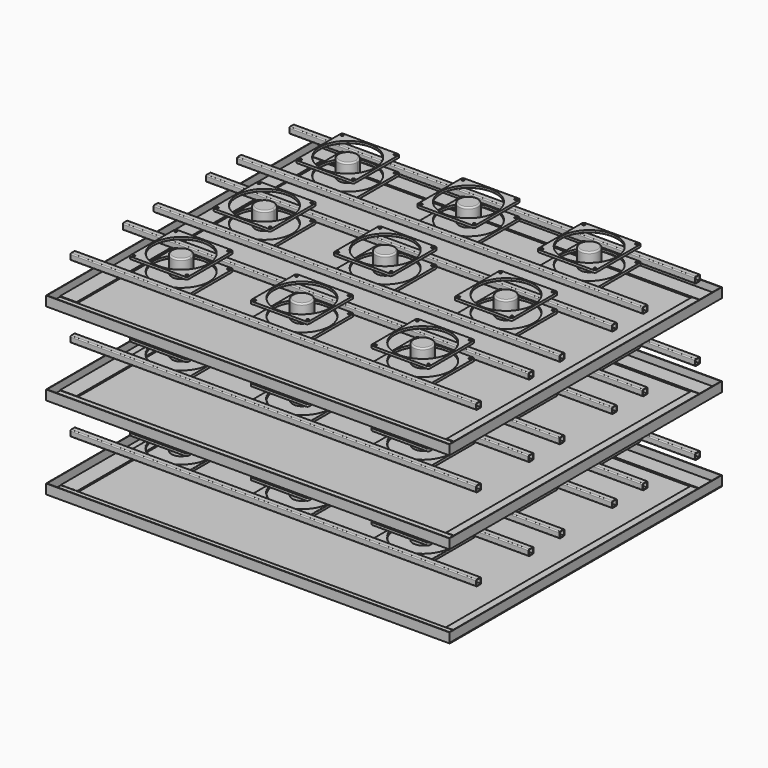
from build123d import *

# Parameters (mm, degrees)
F0_W      = 835
F0_H      = 705
F0_W_2    = 833
F0_H_2    = 703
F1_DEPTH  = 20
F2_W      = 833
F2_H      = 703
F3_DEPTH  = 1
F5_DEPTH  = 3
F6_DEPTH  = 3
F8_DEPTH  = 3
F9_DEPTH  = 3
F10_W     = 10.7
F10_H     = 10.7
F11_DEPTH = 840
F10_W_2   = 10.7000157356
F10_H_2   = 10.7000157356
F10_W_3   = 705
F10_H_3   = 20
F13_DEPTH = 38
F14_R     = 3
F12_R     = 2.5
F16_DEPTH = 5
F17_R     = 1
F18_R     = 2.5
F18_R_2   = 57.5
F19_DEPTH = 5
F20_R     = 1
F21_R     = 3
F12_R_2   = 57.5
F23_DEPTH = 5
F25_DEPTH = 5
F12_R_3   = 20
F26_DEPTH = 38
F27_R     = 3
F28_R     = 1
F29_R     = 1
F30_DEPTH = 38
F31_R     = 3
F32_DEPTH = 5
F33_DEPTH = 5
F34_R     = 1
F35_R     = 3
F36_R     = 3
F37_DEPTH = 5
F38_DEPTH = 38
F40_DEPTH = 5
F41_DEPTH = 38
F42_R     = 3
F42_2_R   = 3
F42_3_R   = 3
F42_4_R   = 3
F42_5_R   = 3
F42_6_R   = 3
F43_R     = 1
F43_2_R   = 1
F43_3_R   = 1
F43_4_R   = 1
F43_5_R   = 1
F43_6_R   = 1
F44_DEPTH = 5
F45_R     = 1
F45_2_R   = 1
F45_3_R   = 1
F45_4_R   = 1
F45_5_R   = 1
F45_6_R   = 1
F46_DEPTH = 5
F47_W     = 833
F47_H     = 703
F48_DEPTH = 18
F50_DEPTH = 3
F51_DEPTH = 3
F52_DEPTH = 5
F53_W     = 833
F53_H     = 703
F54_DEPTH = 18
F56_DEPTH = 3
F58_DEPTH = 38
F57_R     = 20
F57_R_2   = 2.5
F60_DEPTH = 5
F57_R_3   = 57.5
F61_R     = 3
F61_2_R   = 3
F61_3_R   = 3
F61_4_R   = 3
F61_5_R   = 3
F61_6_R   = 3
F61_7_R   = 3
F61_8_R   = 3
F61_9_R   = 3
F62_R     = 1
F62_2_R   = 1
F62_3_R   = 1
F62_4_R   = 1
F62_5_R   = 1
F62_6_R   = 1
F62_7_R   = 1
F62_8_R   = 1
F62_9_R   = 1
F63_R     = 2.5
F63_R_2   = 57.5
F64_DEPTH = 5
F65_R     = 3
F65_2_R   = 3
F65_3_R   = 3
F65_4_R   = 3
F65_5_R   = 3
F65_6_R   = 3
F65_7_R   = 3
F65_8_R   = 3
F65_9_R   = 3
F66_R     = 1
F66_2_R   = 1
F66_3_R   = 1
F66_4_R   = 1
F66_5_R   = 1
F66_6_R   = 1
F66_7_R   = 1
F66_8_R   = 1
F66_9_R   = 1
F67_R     = 2.5
F68_DEPTH = 5
F67_R_2   = 57.5
F70_DEPTH = 38
F67_R_3   = 20
F71_R     = 3
F71_2_R   = 3
F71_3_R   = 3
F71_4_R   = 3
F71_5_R   = 3
F71_6_R   = 3
F71_7_R   = 3
F71_8_R   = 3
F71_9_R   = 3
F72_R     = 1
F72_2_R   = 1
F72_3_R   = 1
F72_4_R   = 1
F72_5_R   = 1
F72_6_R   = 1
F72_7_R   = 1
F72_8_R   = 1
F72_9_R   = 1
F73_R     = 2.5
F73_R_2   = 57.5
F74_DEPTH = 5
F75_R     = 3
F75_2_R   = 3
F75_3_R   = 3
F75_4_R   = 3
F75_5_R   = 3
F75_6_R   = 3
F75_7_R   = 3
F75_8_R   = 3
F75_9_R   = 3
F76_R     = 1
F76_2_R   = 1
F76_3_R   = 1
F76_4_R   = 1
F76_5_R   = 1
F76_6_R   = 1
F76_7_R   = 1
F76_8_R   = 1
F76_9_R   = 1


# Not quite as in the source:
# - a feature names something its author has since deleted; it is built from what else it names
# - the program builds the solid bodies; features that only make, move or delete a surface that nothing else refers to are left out


with BuildPart() as f1:
    # F0 (on Top) → F1 (new body)
    with BuildSketch(Plane.XY):
        with Locations((-169.9971160755, 1.7268359661)):
            Rectangle(F0_W, F0_H)
        with Locations((-169.9971160755, 1.7268359661)):
            Rectangle(F0_W_2, F0_H_2, mode=Mode.SUBTRACT)
    extrude(amount=F1_DEPTH)

    # F2 (on Top) → F3 (join)
    with BuildSketch(Plane.XY):
        with Locations((-168.440297246, 1.221115913)):
            Rectangle(F2_W, F2_H)
    extrude(amount=F3_DEPTH)


with BuildPart() as f5:
    # F4 (on face) → F5 (new body)
    with BuildSketch(Plane.XY.offset(1)):
        Polygon((245.7812933393, 352.721115913), (-169.2187066607, 352.721115913), (-584.2187066607, 352.721115913), (-584.2187066607, 319.721115913), (-169.2187066607, 319.721115913), (245.7812933393, 319.721115913), align=None)
    extrude(amount=F5_DEPTH)


with BuildPart() as f6:
    # F4 (on face) → F6 (new body)
    with BuildSketch(Plane.XY.offset(1)):
        Polygon((-584.2187066607, -316.7731640339), (-584.2187066607, -349.7731640339), (-169.2187066607, -349.7731640339), (245.7812933393, -349.7731640339), (245.7812933393, -316.7731640339), (-169.2187066607, -316.7731640339), align=None)
    extrude(amount=F6_DEPTH)


with BuildPart() as f8:
    # F7 (on face) → F8 (new body)
    with BuildSketch(Plane.XY.offset(1)):
        Polygon((-550.940297246, 318.9739759395), (-584.940297246, 318.9739759395), (-584.940297246, 1.4739759395), (-584.940297246, -316.0260240605), (-550.940297246, -316.0260240605), (-550.940297246, 1.4739759395), align=None)
    extrude(amount=F8_DEPTH)


with BuildPart() as f8b:
    # F7 (on face) → F8, piece 2 (new body)
    with BuildSketch(Plane.XY.offset(1)):
        Polygon((246.5028839245, 1.4739759395), (246.5028839245, 317.5), (212.5028839245, 317.5), (212.5028839245, 1.4739759395), (212.5028839245, 0), (212.5028839245, -316.0260240605), (246.5028839245, -316.0260240605), (246.5028839245, 0), align=None)
    extrude(amount=F8_DEPTH)


with BuildPart() as f9:
    # F7 (on face) → F9 (new body)
    with BuildSketch(Plane.XY.offset(1)):
        Polygon((246.5028839245, 1.4739759395), (246.5028839245, 317.5), (212.5028839245, 317.5), (212.5028839245, 1.4739759395), (212.5028839245, 0), (212.5028839245, -316.0260240605), (246.5028839245, -316.0260240605), (246.5028839245, 0), align=None)
    extrude(amount=F9_DEPTH)


with BuildPart() as f11:
    # F10 (on face) → F11 (new body)
    with BuildSketch(Plane(origin=(-587.4971160755, 0, 0), x_dir=(0, -1, 0), z_dir=(-1, 0, 0))):
        with BuildLine():
            Line((277.1731640339, 79.3), (285.8731640339, 79.3))
            ThreePointArc((285.8731640339, 79.3), (287.2873775963, 79.8857864376), (287.8731640339, 81.3))
            Line((287.8731640339, 81.3), (287.8731640339, 90))
            ThreePointArc((287.8731640339, 90), (287.2873775963, 91.4142135624), (285.8731640339, 92))
            Line((285.8731640339, 92), (277.1731640339, 92))
            ThreePointArc((277.1731640339, 92), (275.7589504715, 91.4142135624), (275.1731640339, 90))
            Line((275.1731640339, 90), (275.1731640339, 81.3))
            ThreePointArc((275.1731640339, 81.3), (275.7589504715, 79.8857864376), (277.1731640339, 79.3))
        make_face()
        with Locations((281.5231640339, 85.65)):
            Rectangle(F10_W, F10_H, mode=Mode.SUBTRACT)
    extrude(amount=-F11_DEPTH)


with BuildPart() as f11b:
    # F10 (on face) → F11, piece 2 (new body)
    with BuildSketch(Plane(origin=(-587.4971160755, 0, 0), x_dir=(0, -1, 0), z_dir=(-1, 0, 0))):
        with BuildLine():
            Line((141.4731640339, 79.3), (150.1731640339, 79.3))
            ThreePointArc((150.1731640339, 79.3), (151.5873775963, 79.8857864376), (152.1731640339, 81.3))
            Line((152.1731640339, 81.3), (152.1731640339, 90))
            ThreePointArc((152.1731640339, 90), (151.5873775963, 91.4142135624), (150.1731640339, 92))
            Line((150.1731640339, 92), (141.4731640339, 92))
            ThreePointArc((141.4731640339, 92), (140.0589504715, 91.4142135624), (139.4731640339, 90))
            Line((139.4731640339, 90), (139.4731640339, 81.3))
            ThreePointArc((139.4731640339, 81.3), (140.0589504715, 79.8857864376), (141.4731640339, 79.3))
        make_face()
        with Locations((145.8231640339, 85.65)):
            Rectangle(F10_W, F10_H, mode=Mode.SUBTRACT)
    extrude(amount=-F11_DEPTH)


with BuildPart() as f11c:
    # F10 (on face) → F11, piece 3 (new body)
    with BuildSketch(Plane(origin=(-587.4971160755, 0, 0), x_dir=(0, -1, 0), z_dir=(-1, 0, 0))):
        with BuildLine():
            Line((61.7731640339, 79.3), (70.4731640339, 79.3))
            ThreePointArc((70.4731640339, 79.3), (71.8873775963, 79.8857864376), (72.4731640339, 81.3))
            Line((72.4731640339, 81.3), (72.4731640339, 90))
            ThreePointArc((72.4731640339, 90), (71.8873775963, 91.4142135624), (70.4731640339, 92))
            Line((70.4731640339, 92), (61.7731640339, 92))
            ThreePointArc((61.7731640339, 92), (60.3589504715, 91.4142135624), (59.7731640339, 90))
            Line((59.7731640339, 90), (59.7731640339, 81.3))
            ThreePointArc((59.7731640339, 81.3), (60.3589504715, 79.8857864376), (61.7731640339, 79.3))
        make_face()
        with Locations((66.1231640339, 85.65)):
            Rectangle(F10_W, F10_H, mode=Mode.SUBTRACT)
    extrude(amount=-F11_DEPTH)


with BuildPart() as f11d:
    # F10 (on face) → F11, piece 4 (new body)
    with BuildSketch(Plane(origin=(-587.4971160755, 0, 0), x_dir=(0, -1, 0), z_dir=(-1, 0, 0))):
        with BuildLine():
            Line((-73.9268359661, 79.3), (-65.2268359661, 79.3))
            ThreePointArc((-65.2268359661, 79.3), (-63.8126224037, 79.8857864376), (-63.2268359661, 81.3))
            Line((-63.2268359661, 81.3), (-63.2268359661, 90))
            ThreePointArc((-63.2268359661, 90), (-63.8126224037, 91.4142135624), (-65.2268359661, 92))
            Line((-65.2268359661, 92), (-73.9268359661, 92))
            ThreePointArc((-73.9268359661, 92), (-75.3410495285, 91.4142135624), (-75.9268359661, 90))
            Line((-75.9268359661, 90), (-75.9268359661, 81.3))
            ThreePointArc((-75.9268359661, 81.3), (-75.3410495285, 79.8857864376), (-73.9268359661, 79.3))
        make_face()
        with Locations((-69.5768359661, 85.65)):
            Rectangle(F10_W, F10_H, mode=Mode.SUBTRACT)
    extrude(amount=-F11_DEPTH)


with BuildPart() as f11e:
    # F10 (on face) → F11, piece 5 (new body)
    with BuildSketch(Plane(origin=(-587.4971160755, 0, 0), x_dir=(0, -1, 0), z_dir=(-1, 0, 0))):
        with BuildLine():
            Line((-153.6268359661, 79.3), (-144.9268359661, 79.3))
            ThreePointArc((-144.9268359661, 79.3), (-143.5126224037, 79.8857864376), (-142.9268359661, 81.3))
            Line((-142.9268359661, 81.3), (-142.9268359661, 90))
            ThreePointArc((-142.9268359661, 90), (-143.5126224037, 91.4142135624), (-144.9268359661, 92))
            Line((-144.9268359661, 92), (-153.6268359661, 92))
            ThreePointArc((-153.6268359661, 92), (-155.0410495285, 91.4142135624), (-155.6268359661, 90))
            Line((-155.6268359661, 90), (-155.6268359661, 81.3))
            ThreePointArc((-155.6268359661, 81.3), (-155.0410495285, 79.8857864376), (-153.6268359661, 79.3))
        make_face()
        with Locations((-149.2768359661, 85.65)):
            Rectangle(F10_W, F10_H, mode=Mode.SUBTRACT)
    extrude(amount=-F11_DEPTH)


with BuildPart() as f11f:
    # F10 (on face) → F11, piece 6 (new body)
    with BuildSketch(Plane(origin=(-587.4971160755, 0, 0), x_dir=(0, -1, 0), z_dir=(-1, 0, 0))):
        with BuildLine():
            Line((-289.3268359661, 79.3), (-280.6268359661, 79.3))
            ThreePointArc((-280.6268359661, 79.3), (-279.2126224037, 79.8857864376), (-278.6268359661, 81.3))
            Line((-278.6268359661, 81.3), (-278.6268359661, 90))
            ThreePointArc((-278.6268359661, 90), (-279.2126224037, 91.4142135624), (-280.6268359661, 92))
            Line((-280.6268359661, 92), (-289.3268359661, 92))
            ThreePointArc((-289.3268359661, 92), (-290.7410495285, 91.4142135624), (-291.3268359661, 90))
            Line((-291.3268359661, 90), (-291.3268359661, 81.3))
            ThreePointArc((-291.3268359661, 81.3), (-290.7410495285, 79.8857864376), (-289.3268359661, 79.3))
        make_face()
        with Locations((-284.9768359661, 85.65)):
            Rectangle(F10_W_2, F10_H_2, mode=Mode.SUBTRACT)
    extrude(amount=-F11_DEPTH)


with BuildPart() as f11g:
    # F10 (on face) → F11, piece 7 (new body)
    with BuildSketch(Plane(origin=(-587.4971160755, 0, 0), x_dir=(0, -1, 0), z_dir=(-1, 0, 0))):
        with BuildLine():
            Line((277.1731640339, 250.6), (285.8731640339, 250.6))
            ThreePointArc((285.8731640339, 250.6), (287.2873775963, 251.1857864376), (287.8731640339, 252.6))
            Line((287.8731640339, 252.6), (287.8731640339, 261.3))
            ThreePointArc((287.8731640339, 261.3), (287.2873775963, 262.7142135624), (285.8731640339, 263.3))
            Line((285.8731640339, 263.3), (277.1731640339, 263.3))
            ThreePointArc((277.1731640339, 263.3), (275.7589504715, 262.7142135624), (275.1731640339, 261.3))
            Line((275.1731640339, 261.3), (275.1731640339, 252.6))
            ThreePointArc((275.1731640339, 252.6), (275.7589504715, 251.1857864376), (277.1731640339, 250.6))
        make_face()
        with Locations((281.5231640339, 256.95)):
            Rectangle(F10_W, F10_H, mode=Mode.SUBTRACT)
    extrude(amount=-F11_DEPTH)


with BuildPart() as f11h:
    # F10 (on face) → F11, piece 8 (new body)
    with BuildSketch(Plane(origin=(-587.4971160755, 0, 0), x_dir=(0, -1, 0), z_dir=(-1, 0, 0))):
        with BuildLine():
            Line((141.4731640339, 250.6), (150.1731640339, 250.6))
            ThreePointArc((150.1731640339, 250.6), (151.5873775963, 251.1857864376), (152.1731640339, 252.6))
            Line((152.1731640339, 252.6), (152.1731640339, 261.3))
            ThreePointArc((152.1731640339, 261.3), (151.5873775963, 262.7142135624), (150.1731640339, 263.3))
            Line((150.1731640339, 263.3), (141.4731640339, 263.3))
            ThreePointArc((141.4731640339, 263.3), (140.0589504715, 262.7142135624), (139.4731640339, 261.3))
            Line((139.4731640339, 261.3), (139.4731640339, 252.6))
            ThreePointArc((139.4731640339, 252.6), (140.0589504715, 251.1857864376), (141.4731640339, 250.6))
        make_face()
        with Locations((145.8231640339, 256.95)):
            Rectangle(F10_W, F10_H, mode=Mode.SUBTRACT)
    extrude(amount=-F11_DEPTH)


with BuildPart() as f11i:
    # F10 (on face) → F11, piece 9 (new body)
    with BuildSketch(Plane(origin=(-587.4971160755, 0, 0), x_dir=(0, -1, 0), z_dir=(-1, 0, 0))):
        with BuildLine():
            Line((61.7731640339, 250.6), (70.4731640339, 250.6))
            ThreePointArc((70.4731640339, 250.6), (71.8873775963, 251.1857864376), (72.4731640339, 252.6))
            Line((72.4731640339, 252.6), (72.4731640339, 261.3))
            ThreePointArc((72.4731640339, 261.3), (71.8873775963, 262.7142135624), (70.4731640339, 263.3))
            Line((70.4731640339, 263.3), (61.7731640339, 263.3))
            ThreePointArc((61.7731640339, 263.3), (60.3589504715, 262.7142135624), (59.7731640339, 261.3))
            Line((59.7731640339, 261.3), (59.7731640339, 252.6))
            ThreePointArc((59.7731640339, 252.6), (60.3589504715, 251.1857864376), (61.7731640339, 250.6))
        make_face()
        with Locations((66.1231640339, 256.95)):
            Rectangle(F10_W, F10_H, mode=Mode.SUBTRACT)
    extrude(amount=-F11_DEPTH)


with BuildPart() as f11j:
    # F10 (on face) → F11, piece 10 (new body)
    with BuildSketch(Plane(origin=(-587.4971160755, 0, 0), x_dir=(0, -1, 0), z_dir=(-1, 0, 0))):
        with BuildLine():
            Line((-73.9268359661, 250.6), (-65.2268359661, 250.6))
            ThreePointArc((-65.2268359661, 250.6), (-63.8126224037, 251.1857864376), (-63.2268359661, 252.6))
            Line((-63.2268359661, 252.6), (-63.2268359661, 261.3))
            ThreePointArc((-63.2268359661, 261.3), (-63.8126224037, 262.7142135624), (-65.2268359661, 263.3))
            Line((-65.2268359661, 263.3), (-73.9268359661, 263.3))
            ThreePointArc((-73.9268359661, 263.3), (-75.3410495285, 262.7142135624), (-75.9268359661, 261.3))
            Line((-75.9268359661, 261.3), (-75.9268359661, 252.6))
            ThreePointArc((-75.9268359661, 252.6), (-75.3410495285, 251.1857864376), (-73.9268359661, 250.6))
        make_face()
        with Locations((-69.5768359661, 256.95)):
            Rectangle(F10_W, F10_H, mode=Mode.SUBTRACT)
    extrude(amount=-F11_DEPTH)


with BuildPart() as f11k:
    # F10 (on face) → F11, piece 11 (new body)
    with BuildSketch(Plane(origin=(-587.4971160755, 0, 0), x_dir=(0, -1, 0), z_dir=(-1, 0, 0))):
        with BuildLine():
            Line((-153.6268359661, 250.6), (-144.9268359661, 250.6))
            ThreePointArc((-144.9268359661, 250.6), (-143.5126224037, 251.1857864376), (-142.9268359661, 252.6))
            Line((-142.9268359661, 252.6), (-142.9268359661, 261.3))
            ThreePointArc((-142.9268359661, 261.3), (-143.5126224037, 262.7142135624), (-144.9268359661, 263.3))
            Line((-144.9268359661, 263.3), (-153.6268359661, 263.3))
            ThreePointArc((-153.6268359661, 263.3), (-155.0410495285, 262.7142135624), (-155.6268359661, 261.3))
            Line((-155.6268359661, 261.3), (-155.6268359661, 252.6))
            ThreePointArc((-155.6268359661, 252.6), (-155.0410495285, 251.1857864376), (-153.6268359661, 250.6))
        make_face()
        with Locations((-149.2768359661, 256.95)):
            Rectangle(F10_W, F10_H, mode=Mode.SUBTRACT)
    extrude(amount=-F11_DEPTH)


with BuildPart() as f11l:
    # F10 (on face) → F11, piece 12 (new body)
    with BuildSketch(Plane(origin=(-587.4971160755, 0, 0), x_dir=(0, -1, 0), z_dir=(-1, 0, 0))):
        with BuildLine():
            Line((-289.3268359661, 250.6), (-280.6268359661, 250.6))
            ThreePointArc((-280.6268359661, 250.6), (-279.2126224037, 251.1857864376), (-278.6268359661, 252.6))
            Line((-278.6268359661, 252.6), (-278.6268359661, 261.3))
            ThreePointArc((-278.6268359661, 261.3), (-279.2126224037, 262.7142135624), (-280.6268359661, 263.3))
            Line((-280.6268359661, 263.3), (-289.3268359661, 263.3))
            ThreePointArc((-289.3268359661, 263.3), (-290.7410495285, 262.7142135624), (-291.3268359661, 261.3))
            Line((-291.3268359661, 261.3), (-291.3268359661, 252.6))
            ThreePointArc((-291.3268359661, 252.6), (-290.7410495285, 251.1857864376), (-289.3268359661, 250.6))
        make_face()
        with Locations((-284.9768359661, 256.95)):
            Rectangle(F10_W_2, F10_H_2, mode=Mode.SUBTRACT)
    extrude(amount=-F11_DEPTH)


with BuildPart() as f11m:
    # F10 (on face) → F11, piece 13 (new body)
    with BuildSketch(Plane(origin=(-587.4971160755, 0, 0), x_dir=(0, -1, 0), z_dir=(-1, 0, 0))):
        with BuildLine():
            Line((277.1731640339, 400.917163891), (285.8731640339, 400.917163891))
            ThreePointArc((285.8731640339, 400.917163891), (287.2873775963, 401.5029503286), (287.8731640339, 402.917163891))
            Line((287.8731640339, 402.917163891), (287.8731640339, 411.617163891))
            ThreePointArc((287.8731640339, 411.617163891), (287.2873775963, 413.0313774534), (285.8731640339, 413.617163891))
            Line((285.8731640339, 413.617163891), (277.1731640339, 413.617163891))
            ThreePointArc((277.1731640339, 413.617163891), (275.7589504715, 413.0313774534), (275.1731640339, 411.617163891))
            Line((275.1731640339, 411.617163891), (275.1731640339, 402.917163891))
            ThreePointArc((275.1731640339, 402.917163891), (275.7589504715, 401.5029503286), (277.1731640339, 400.917163891))
        make_face()
        with Locations((281.5231640339, 407.267163891)):
            Rectangle(F10_W, F10_H, mode=Mode.SUBTRACT)
    extrude(amount=-F11_DEPTH)


with BuildPart() as f11n:
    # F10 (on face) → F11, piece 14 (new body)
    with BuildSketch(Plane(origin=(-587.4971160755, 0, 0), x_dir=(0, -1, 0), z_dir=(-1, 0, 0))):
        with BuildLine():
            Line((141.4731640339, 400.917163891), (150.1731640339, 400.917163891))
            ThreePointArc((150.1731640339, 400.917163891), (151.5873775963, 401.5029503286), (152.1731640339, 402.917163891))
            Line((152.1731640339, 402.917163891), (152.1731640339, 411.617163891))
            ThreePointArc((152.1731640339, 411.617163891), (151.5873775963, 413.0313774534), (150.1731640339, 413.617163891))
            Line((150.1731640339, 413.617163891), (141.4731640339, 413.617163891))
            ThreePointArc((141.4731640339, 413.617163891), (140.0589504715, 413.0313774534), (139.4731640339, 411.617163891))
            Line((139.4731640339, 411.617163891), (139.4731640339, 402.917163891))
            ThreePointArc((139.4731640339, 402.917163891), (140.0589504715, 401.5029503286), (141.4731640339, 400.917163891))
        make_face()
        with Locations((145.8231640339, 407.267163891)):
            Rectangle(F10_W, F10_H, mode=Mode.SUBTRACT)
    extrude(amount=-F11_DEPTH)


with BuildPart() as f11o:
    # F10 (on face) → F11, piece 15 (new body)
    with BuildSketch(Plane(origin=(-587.4971160755, 0, 0), x_dir=(0, -1, 0), z_dir=(-1, 0, 0))):
        with BuildLine():
            Line((61.7731640339, 400.917163891), (70.4731640339, 400.917163891))
            ThreePointArc((70.4731640339, 400.917163891), (71.8873775963, 401.5029503286), (72.4731640339, 402.917163891))
            Line((72.4731640339, 402.917163891), (72.4731640339, 411.617163891))
            ThreePointArc((72.4731640339, 411.617163891), (71.8873775963, 413.0313774534), (70.4731640339, 413.617163891))
            Line((70.4731640339, 413.617163891), (61.7731640339, 413.617163891))
            ThreePointArc((61.7731640339, 413.617163891), (60.3589504715, 413.0313774534), (59.7731640339, 411.617163891))
            Line((59.7731640339, 411.617163891), (59.7731640339, 402.917163891))
            ThreePointArc((59.7731640339, 402.917163891), (60.3589504715, 401.5029503286), (61.7731640339, 400.917163891))
        make_face()
        with Locations((66.1231640339, 407.267163891)):
            Rectangle(F10_W, F10_H, mode=Mode.SUBTRACT)
    extrude(amount=-F11_DEPTH)


with BuildPart() as f11p:
    # F10 (on face) → F11, piece 16 (new body)
    with BuildSketch(Plane(origin=(-587.4971160755, 0, 0), x_dir=(0, -1, 0), z_dir=(-1, 0, 0))):
        with BuildLine():
            Line((-73.9268359661, 400.917163891), (-65.2268359661, 400.917163891))
            ThreePointArc((-65.2268359661, 400.917163891), (-63.8126224037, 401.5029503286), (-63.2268359661, 402.917163891))
            Line((-63.2268359661, 402.917163891), (-63.2268359661, 411.617163891))
            ThreePointArc((-63.2268359661, 411.617163891), (-63.8126224037, 413.0313774534), (-65.2268359661, 413.617163891))
            Line((-65.2268359661, 413.617163891), (-73.9268359661, 413.617163891))
            ThreePointArc((-73.9268359661, 413.617163891), (-75.3410495285, 413.0313774534), (-75.9268359661, 411.617163891))
            Line((-75.9268359661, 411.617163891), (-75.9268359661, 402.917163891))
            ThreePointArc((-75.9268359661, 402.917163891), (-75.3410495285, 401.5029503286), (-73.9268359661, 400.917163891))
        make_face()
        with Locations((-69.5768359661, 407.267163891)):
            Rectangle(F10_W, F10_H, mode=Mode.SUBTRACT)
    extrude(amount=-F11_DEPTH)


with BuildPart() as f11q:
    # F10 (on face) → F11, piece 17 (new body)
    with BuildSketch(Plane(origin=(-587.4971160755, 0, 0), x_dir=(0, -1, 0), z_dir=(-1, 0, 0))):
        with BuildLine():
            Line((-153.6268359661, 400.917163891), (-144.9268359661, 400.917163891))
            ThreePointArc((-144.9268359661, 400.917163891), (-143.5126224037, 401.5029503286), (-142.9268359661, 402.917163891))
            Line((-142.9268359661, 402.917163891), (-142.9268359661, 411.617163891))
            ThreePointArc((-142.9268359661, 411.617163891), (-143.5126224037, 413.0313774534), (-144.9268359661, 413.617163891))
            Line((-144.9268359661, 413.617163891), (-153.6268359661, 413.617163891))
            ThreePointArc((-153.6268359661, 413.617163891), (-155.0410495285, 413.0313774534), (-155.6268359661, 411.617163891))
            Line((-155.6268359661, 411.617163891), (-155.6268359661, 402.917163891))
            ThreePointArc((-155.6268359661, 402.917163891), (-155.0410495285, 401.5029503286), (-153.6268359661, 400.917163891))
        make_face()
        with Locations((-149.2768359661, 407.267163891)):
            Rectangle(F10_W, F10_H, mode=Mode.SUBTRACT)
    extrude(amount=-F11_DEPTH)


with BuildPart() as f11r:
    # F10 (on face) → F11, piece 18 (new body)
    with BuildSketch(Plane(origin=(-587.4971160755, 0, 0), x_dir=(0, -1, 0), z_dir=(-1, 0, 0))):
        with BuildLine():
            Line((-289.3268359661, 400.917163891), (-280.6268359661, 400.917163891))
            ThreePointArc((-280.6268359661, 400.917163891), (-279.2126224037, 401.5029503286), (-278.6268359661, 402.917163891))
            Line((-278.6268359661, 402.917163891), (-278.6268359661, 411.617163891))
            ThreePointArc((-278.6268359661, 411.617163891), (-279.2126224037, 413.0313774534), (-280.6268359661, 413.617163891))
            Line((-280.6268359661, 413.617163891), (-289.3268359661, 413.617163891))
            ThreePointArc((-289.3268359661, 413.617163891), (-290.7410495285, 413.0313774534), (-291.3268359661, 411.617163891))
            Line((-291.3268359661, 411.617163891), (-291.3268359661, 402.917163891))
            ThreePointArc((-291.3268359661, 402.917163891), (-290.7410495285, 401.5029503286), (-289.3268359661, 400.917163891))
        make_face()
        with Locations((-284.9768359661, 407.267163891)):
            Rectangle(F10_W_2, F10_H_2, mode=Mode.SUBTRACT)
    extrude(amount=-F11_DEPTH)


with BuildPart() as f11s:
    # F10 (on face) → F11, piece 19 (new body)
    with BuildSketch(Plane(origin=(-587.4971160755, 0, 0), x_dir=(0, -1, 0), z_dir=(-1, 0, 0))):
        with Locations((-1.7268359661, 181.3)):
            Rectangle(F10_W_3, F10_H_3)
    extrude(amount=-F11_DEPTH)

    # F46 (cut): a face of the model
    f46_faces = [f11s.faces().sort_by_distance(p)[0] for p in [
        (252.5028839245, 1.7268359661, 181.3),
    ]]
    extrude(f46_faces, amount=-F46_DEPTH, mode=Mode.SUBTRACT)

    # F47 (on face) → F48 (cut)
    with BuildSketch(Plane.XY.offset(191.3)):
        with Locations((-169.9971160755, 1.7268359661)):
            Rectangle(F47_W, F47_H)
    extrude(amount=-F48_DEPTH, mode=Mode.SUBTRACT)


with BuildPart() as f11t:
    # F10 (on face) → F11, piece 20 (new body)
    with BuildSketch(Plane(origin=(-587.4971160755, 0, 0), x_dir=(0, -1, 0), z_dir=(-1, 0, 0))):
        with Locations((-1.7268359661, 352.6)):
            Rectangle(F10_W_3, F10_H_3)
    extrude(amount=-F11_DEPTH)

    # F52 (cut): a face of the model
    f52_faces = [f11t.faces().sort_by_distance(p)[0] for p in [
        (252.5028839245, 1.7268359661, 352.6),
    ]]
    extrude(f52_faces, amount=-F52_DEPTH, mode=Mode.SUBTRACT)

    # F53 (on face) → F54 (cut)
    with BuildSketch(Plane.XY.offset(362.6)):
        with Locations((-169.9971160755, 1.7268359661)):
            Rectangle(F53_W, F53_H)
    extrude(amount=-F54_DEPTH, mode=Mode.SUBTRACT)


with BuildPart() as f13:
    # F12 (on face) → F13 (new body)
    with BuildSketch(Plane(origin=(0, 0, 79.3), x_dir=(1, 0, 0), z_dir=(0, 0, -1))):
        with BuildLine():
            ThreePointArc((-397.4971160755, -217.1268359661), (-431.6392516992, -202.9847003424), (-417.4971160755, -237.1268359661))
            ThreePointArc((-417.4971160755, -237.1268359661), (-403.3549804517, -231.2689715898), (-397.4971160755, -217.1268359661))
        make_face()
    extrude(amount=-F13_DEPTH)

    # F14
    f14_edges = [f13.edges().sort_by_distance(p)[0] for p in [
        (-417.497116, 197.126836, 79.3),
    ]]
    fillet(f14_edges, radius=F14_R)

    # F21
    f21_edges = [f13.edges().sort_by_distance(p)[0] for p in [
        (-417.497116, 197.126836, 117.3),
    ]]
    fillet(f21_edges, radius=F21_R)


with BuildPart() as f16:
    # F12 (on face) → F16 (new body)
    with BuildSketch(Plane(origin=(0, 0, 79.3), x_dir=(1, 0, 0), z_dir=(0, 0, -1))):
        with BuildLine():
            Line((-473.4971160755, -277.1268359661), (-417.4971160755, -277.1268359661))
            Line((-417.4971160755, -277.1268359661), (-361.4971160755, -277.1268359661))
            ThreePointArc((-361.4971160755, -277.1268359661), (-358.6686889507, -275.9552630909), (-357.4971160755, -273.1268359661))
            Line((-357.4971160755, -273.1268359661), (-357.4971160755, -161.1268359661))
            ThreePointArc((-357.4971160755, -161.1268359661), (-358.6686889507, -158.2984088414), (-361.4971160755, -157.1268359661))
            Line((-361.4971160755, -157.1268359661), (-473.4971160755, -157.1268359661))
            ThreePointArc((-473.4971160755, -157.1268359661), (-476.3255432002, -158.2984088414), (-477.4971160755, -161.1268359661))
            Line((-477.4971160755, -161.1268359661), (-477.4971160755, -273.1268359661))
            ThreePointArc((-477.4971160755, -273.1268359661), (-476.3255432002, -275.9552630909), (-473.4971160755, -277.1268359661))
        make_face()
        with Locations((-471.8496011495, -271.2464916975)):
            Circle(F12_R, mode=Mode.SUBTRACT)
        with BuildLine():
            ThreePointArc((-359.9971160755, -217.1268359661), (-376.8384761572, -257.7854758843), (-417.4971160755, -274.6268359661))
            ThreePointArc((-417.4971160755, -274.6268359661), (-458.1557559937, -176.4681960479), (-359.9971160755, -217.1268359661))
        make_face(mode=Mode.SUBTRACT)
        with Locations((-471.6119623187, -162.7688455012)):
            Circle(F12_R, mode=Mode.SUBTRACT)
        with Locations((-362.9982335222, -271.1276745391)):
            Circle(F12_R, mode=Mode.SUBTRACT)
        with Locations((-362.6935253453, -163.3219680485)):
            Circle(F12_R, mode=Mode.SUBTRACT)
    extrude(amount=-F16_DEPTH)

    # F17
    f17_edges = [f16.edges().sort_by_distance(p)[0] for p in [
        (-474.997116, 217.126836, 79.3),
    ]]
    fillet(f17_edges, radius=F17_R)


with BuildPart() as f19:
    # F18 (on face) → F19 (new body)
    with BuildSketch(Plane.XY.offset(117.3)):
        with BuildLine():
            Line((-473.4971160755, 157.1268359661), (-361.4971160755, 157.1268359661))
            ThreePointArc((-361.4971160755, 157.1268359661), (-358.6686889507, 158.2984088414), (-357.4971160755, 161.1268359661))
            Line((-357.4971160755, 161.1268359661), (-357.4971160755, 273.1268359661))
            ThreePointArc((-357.4971160755, 273.1268359661), (-358.6686889507, 275.9552630909), (-361.4971160755, 277.1268359661))
            Line((-361.4971160755, 277.1268359661), (-473.4971160755, 277.1268359661))
            ThreePointArc((-473.4971160755, 277.1268359661), (-476.3255432002, 275.9552630909), (-477.4971160755, 273.1268359661))
            Line((-477.4971160755, 273.1268359661), (-477.4971160755, 161.1268359661))
            ThreePointArc((-477.4971160755, 161.1268359661), (-476.3255432002, 158.2984088414), (-473.4971160755, 157.1268359661))
        make_face()
        with Locations((-471.8734597501, 163.0278199579)):
            Circle(F18_R, mode=Mode.SUBTRACT)
        with Locations((-362.4497238937, 163.4382291271)):
            Circle(F18_R, mode=Mode.SUBTRACT)
        with Locations((-417.4971160755, 217.1268359661)):
            Circle(F18_R_2, mode=Mode.SUBTRACT)
        with Locations((-471.9772779604, 271.1418694415)):
            Circle(F18_R, mode=Mode.SUBTRACT)
        with Locations((-363.4227434503, 271.5324836796)):
            Circle(F18_R, mode=Mode.SUBTRACT)
    extrude(amount=F19_DEPTH)

    # F20
    f20_edges = [f19.edges().sort_by_distance(p)[0] for p in [
        (-474.997116, 217.126836, 122.3),
    ]]
    fillet(f20_edges, radius=F20_R)


with BuildPart() as f23:
    # F12 (on face) → F23 (new body)
    with BuildSketch(Plane(origin=(0, 0, 79.3), x_dir=(1, 0, 0), z_dir=(0, 0, -1))):
        with BuildLine():
            Line((26.5028839245, -277.1268359661), (138.5028839245, -277.1268359661))
            ThreePointArc((138.5028839245, -277.1268359661), (141.3313110493, -275.9552630909), (142.5028839245, -273.1268359661))
            Line((142.5028839245, -273.1268359661), (142.5028839245, -161.1268359661))
            ThreePointArc((142.5028839245, -161.1268359661), (141.3313110493, -158.2984088414), (138.5028839245, -157.1268359661))
            Line((138.5028839245, -157.1268359661), (26.5028839245, -157.1268359661))
            ThreePointArc((26.5028839245, -157.1268359661), (23.6744567998, -158.2984088414), (22.5028839245, -161.1268359661))
            Line((22.5028839245, -161.1268359661), (22.5028839245, -273.1268359661))
            ThreePointArc((22.5028839245, -273.1268359661), (23.6744567998, -275.9552630909), (26.5028839245, -277.1268359661))
        make_face()
        with Locations((28.1503988505, -271.2464916975)):
            Circle(F12_R, mode=Mode.SUBTRACT)
        with Locations((28.3880376813, -162.7688455012)):
            Circle(F12_R, mode=Mode.SUBTRACT)
        with Locations((137.0017664778, -271.1276745391)):
            Circle(F12_R, mode=Mode.SUBTRACT)
        with Locations((82.5028839245, -217.1268359661)):
            Circle(F12_R_2, mode=Mode.SUBTRACT)
        with Locations((137.3064746547, -163.3219680485)):
            Circle(F12_R, mode=Mode.SUBTRACT)
    extrude(amount=-F23_DEPTH)

    # F29
    f29_edges = [f23.edges().sort_by_distance(p)[0] for p in [
        (25.002884, 217.126836, 79.3),
    ]]
    fillet(f29_edges, radius=F29_R)


with BuildPart() as f25:
    # F12 (on face) → F25 (new body)
    with BuildSketch(Plane(origin=(0, 0, 79.3), x_dir=(1, 0, 0), z_dir=(0, 0, -1))):
        with BuildLine():
            Line((-223.4971160755, -277.1268359661), (-111.4971160755, -277.1268359661))
            ThreePointArc((-111.4971160755, -277.1268359661), (-108.6686889507, -275.9552630909), (-107.4971160755, -273.1268359661))
            Line((-107.4971160755, -273.1268359661), (-107.4971160755, -161.1268359661))
            ThreePointArc((-107.4971160755, -161.1268359661), (-108.6686889507, -158.2984088414), (-111.4971160755, -157.1268359661))
            Line((-111.4971160755, -157.1268359661), (-223.4971160755, -157.1268359661))
            ThreePointArc((-223.4971160755, -157.1268359661), (-226.3255432002, -158.2984088414), (-227.4971160755, -161.1268359661))
            Line((-227.4971160755, -161.1268359661), (-227.4971160755, -273.1268359661))
            ThreePointArc((-227.4971160755, -273.1268359661), (-226.3255432002, -275.9552630909), (-223.4971160755, -277.1268359661))
        make_face()
        with Locations((-221.8496011495, -271.2464916975)):
            Circle(F12_R, mode=Mode.SUBTRACT)
        with Locations((-221.6119623187, -162.7688455012)):
            Circle(F12_R, mode=Mode.SUBTRACT)
        with Locations((-112.9982335222, -271.1276745391)):
            Circle(F12_R, mode=Mode.SUBTRACT)
        with Locations((-167.4971160755, -217.1268359661)):
            Circle(F12_R_2, mode=Mode.SUBTRACT)
        with Locations((-112.6935253453, -163.3219680485)):
            Circle(F12_R, mode=Mode.SUBTRACT)
    extrude(amount=-F25_DEPTH)

    # F28
    f28_edges = [f25.edges().sort_by_distance(p)[0] for p in [
        (-224.997116, 217.126836, 79.3),
    ]]
    fillet(f28_edges, radius=F28_R)


with BuildPart() as f26:
    # F12 (on face) → F26 (new body)
    with BuildSketch(Plane(origin=(0, 0, 79.3), x_dir=(1, 0, 0), z_dir=(0, 0, -1))):
        with Locations((-167.4971160755, -217.1268359661)):
            Circle(F12_R_3)
    extrude(amount=-F26_DEPTH)

    # F27
    f27_edges = [f26.edges().sort_by_distance(p)[0] for p in [
        (-187.497116, 217.126836, 79.3),
    ]]
    fillet(f27_edges, radius=F27_R)

    # F35
    f35_edges = [f26.edges().sort_by_distance(p)[0] for p in [
        (-187.497116, 217.126836, 117.3),
    ]]
    fillet(f35_edges, radius=F35_R)


with BuildPart() as f30:
    # F12 (on face) → F30 (new body)
    with BuildSketch(Plane(origin=(0, 0, 79.3), x_dir=(1, 0, 0), z_dir=(0, 0, -1))):
        with Locations((82.5028839245, -217.1268359661)):
            Circle(F12_R_3)
    extrude(amount=-F30_DEPTH)

    # F31
    f31_edges = [f30.edges().sort_by_distance(p)[0] for p in [
        (62.502884, 217.126836, 79.3),
    ]]
    fillet(f31_edges, radius=F31_R)

    # F36
    f36_edges = [f30.edges().sort_by_distance(p)[0] for p in [
        (62.502884, 217.126836, 117.3),
    ]]
    fillet(f36_edges, radius=F36_R)


with BuildPart() as f32:
    # F18 (on face) → F32 (new body)
    with BuildSketch(Plane.XY.offset(117.3)):
        with BuildLine():
            Line((-223.4971160755, 157.1268359661), (-111.4971160755, 157.1268359661))
            ThreePointArc((-111.4971160755, 157.1268359661), (-108.6686889507, 158.2984088414), (-107.4971160755, 161.1268359661))
            Line((-107.4971160755, 161.1268359661), (-107.4971160755, 273.1268359661))
            ThreePointArc((-107.4971160755, 273.1268359661), (-108.6686889507, 275.9552630909), (-111.4971160755, 277.1268359661))
            Line((-111.4971160755, 277.1268359661), (-223.4971160755, 277.1268359661))
            ThreePointArc((-223.4971160755, 277.1268359661), (-226.3255432002, 275.9552630909), (-227.4971160755, 273.1268359661))
            Line((-227.4971160755, 273.1268359661), (-227.4971160755, 161.1268359661))
            ThreePointArc((-227.4971160755, 161.1268359661), (-226.3255432002, 158.2984088414), (-223.4971160755, 157.1268359661))
        make_face()
        with Locations((-221.8734597501, 163.0278199579)):
            Circle(F18_R, mode=Mode.SUBTRACT)
        with Locations((-221.9772779604, 271.1418694415)):
            Circle(F18_R, mode=Mode.SUBTRACT)
        with Locations((-112.4497238937, 163.4382291271)):
            Circle(F18_R, mode=Mode.SUBTRACT)
        with Locations((-167.4971160755, 217.1268359661)):
            Circle(F18_R_2, mode=Mode.SUBTRACT)
        with Locations((-113.4227434503, 271.5324836796)):
            Circle(F18_R, mode=Mode.SUBTRACT)
    extrude(amount=-F32_DEPTH)

    # F34
    f34_edges = [f32.edges().sort_by_distance(p)[0] for p in [
        (-224.997116, 217.126836, 117.3),
    ]]
    fillet(f34_edges, radius=F34_R)


with BuildPart() as f33:
    # F18 (on face) → F33 (new body)
    with BuildSketch(Plane.XY.offset(117.3)):
        with BuildLine():
            Line((26.5028839245, 157.1268359661), (138.5028839245, 157.1268359661))
            ThreePointArc((138.5028839245, 157.1268359661), (141.3313110493, 158.2984088414), (142.5028839245, 161.1268359661))
            Line((142.5028839245, 161.1268359661), (142.5028839245, 273.1268359661))
            ThreePointArc((142.5028839245, 273.1268359661), (141.3313110493, 275.9552630909), (138.5028839245, 277.1268359661))
            Line((138.5028839245, 277.1268359661), (26.5028839245, 277.1268359661))
            ThreePointArc((26.5028839245, 277.1268359661), (23.6744567998, 275.9552630909), (22.5028839245, 273.1268359661))
            Line((22.5028839245, 273.1268359661), (22.5028839245, 161.1268359661))
            ThreePointArc((22.5028839245, 161.1268359661), (23.6744567998, 158.2984088414), (26.5028839245, 157.1268359661))
        make_face()
        with Locations((28.1265402499, 163.0278199579)):
            Circle(F18_R, mode=Mode.SUBTRACT)
        with Locations((137.5502761063, 163.4382291271)):
            Circle(F18_R, mode=Mode.SUBTRACT)
        with Locations((28.0227220396, 271.1418694415)):
            Circle(F18_R, mode=Mode.SUBTRACT)
        with Locations((82.5028839245, 217.1268359661)):
            Circle(F18_R_2, mode=Mode.SUBTRACT)
        with Locations((136.5772565497, 271.5324836796)):
            Circle(F18_R, mode=Mode.SUBTRACT)
    extrude(amount=-F33_DEPTH)


with BuildPart() as f37:
    # F12 (on face) → F37 (new body)
    with BuildSketch(Plane(origin=(0, 0, 79.3), x_dir=(1, 0, 0), z_dir=(0, 0, -1))):
        with BuildLine():
            Line((-473.4971160755, -61.7268359661), (-417.4971160755, -61.7268359661))
            Line((-417.4971160755, -61.7268359661), (-361.4971160755, -61.7268359661))
            ThreePointArc((-361.4971160755, -61.7268359661), (-358.6686889507, -60.5552630909), (-357.4971160755, -57.7268359661))
            Line((-357.4971160755, -57.7268359661), (-357.4971160755, 54.2731640339))
            ThreePointArc((-357.4971160755, 54.2731640339), (-358.6686889507, 57.1015911586), (-361.4971160755, 58.2731640339))
            Line((-361.4971160755, 58.2731640339), (-473.4971160755, 58.2731640339))
            ThreePointArc((-473.4971160755, 58.2731640339), (-476.3255432002, 57.1015911586), (-477.4971160755, 54.2731640339))
            Line((-477.4971160755, 54.2731640339), (-477.4971160755, -57.7268359661))
            ThreePointArc((-477.4971160755, -57.7268359661), (-476.3255432002, -60.5552630909), (-473.4971160755, -61.7268359661))
        make_face()
        with Locations((-471.8496011495, -55.8464916975)):
            Circle(F12_R, mode=Mode.SUBTRACT)
        with Locations((-362.9982335222, -55.7276745391)):
            Circle(F12_R, mode=Mode.SUBTRACT)
        with BuildLine():
            ThreePointArc((-359.9971160755, -1.7268359661), (-376.8384761572, -42.3854758843), (-417.4971160755, -59.2268359661))
            ThreePointArc((-417.4971160755, -59.2268359661), (-458.1557559937, 38.9318039521), (-359.9971160755, -1.7268359661))
        make_face(mode=Mode.SUBTRACT)
        with Locations((-471.6119623187, 52.6311544988)):
            Circle(F12_R, mode=Mode.SUBTRACT)
        with Locations((-362.6935253453, 52.0780319515)):
            Circle(F12_R, mode=Mode.SUBTRACT)
    extrude(amount=-F37_DEPTH)

    # F43
    f43_edges = [f37.edges().sort_by_distance(p)[0] for p in [
        (-417.497116, 61.726836, 84.3),
        (-358.668689, 60.555263, 84.3),
        (-357.497116, 1.726836, 84.3),
        (-358.668689, -57.101591, 84.3),
        (-417.497116, -58.273164, 84.3),
        (-476.325543, -57.101591, 84.3),
        (-477.497116, 1.726836, 84.3),
        (-476.325543, 60.555263, 84.3),
        (-474.349601, 55.846492, 84.3),
        (-365.498234, 55.727675, 84.3),
        (-474.997116, 1.726836, 84.3),
        (-474.111962, -52.631154, 84.3),
        (-365.193525, -52.078032, 84.3),
    ]]
    fillet(f43_edges, radius=F43_R)


with BuildPart() as f38:
    # F12 (on face) → F38 (new body)
    with BuildSketch(Plane(origin=(0, 0, 79.3), x_dir=(1, 0, 0), z_dir=(0, 0, -1))):
        with BuildLine():
            ThreePointArc((-397.4971160755, -1.7268359661), (-431.6392516992, 12.4152996576), (-417.4971160755, -21.7268359661))
            ThreePointArc((-417.4971160755, -21.7268359661), (-403.3549804517, -15.8689715898), (-397.4971160755, -1.7268359661))
        make_face()
    extrude(amount=-F38_DEPTH)

    # F42#6
    f42_6_edges = [f38.edges().sort_by_distance(p)[0] for p in [
        (-417.497116, -18.273164, 117.3),
    ]]
    fillet(f42_6_edges, radius=F42_6_R)


with BuildPart() as f40:
    # F12 (on face) → F40 (new body)
    with BuildSketch(Plane(origin=(0, 0, 79.3), x_dir=(1, 0, 0), z_dir=(0, 0, -1))):
        with BuildLine():
            Line((-223.4971160755, -61.7268359661), (-111.4971160755, -61.7268359661))
            ThreePointArc((-111.4971160755, -61.7268359661), (-108.6686889507, -60.5552630909), (-107.4971160755, -57.7268359661))
            Line((-107.4971160755, -57.7268359661), (-107.4971160755, 54.2731640339))
            ThreePointArc((-107.4971160755, 54.2731640339), (-108.6686889507, 57.1015911586), (-111.4971160755, 58.2731640339))
            Line((-111.4971160755, 58.2731640339), (-223.4971160755, 58.2731640339))
            ThreePointArc((-223.4971160755, 58.2731640339), (-226.3255432002, 57.1015911586), (-227.4971160755, 54.2731640339))
            Line((-227.4971160755, 54.2731640339), (-227.4971160755, -57.7268359661))
            ThreePointArc((-227.4971160755, -57.7268359661), (-226.3255432002, -60.5552630909), (-223.4971160755, -61.7268359661))
        make_face()
        with Locations((-221.8496011495, -55.8464916975)):
            Circle(F12_R, mode=Mode.SUBTRACT)
        with Locations((-112.9982335222, -55.7276745391)):
            Circle(F12_R, mode=Mode.SUBTRACT)
        with Locations((-221.6119623187, 52.6311544988)):
            Circle(F12_R, mode=Mode.SUBTRACT)
        with Locations((-167.4971160755, -1.7268359661)):
            Circle(F12_R_2, mode=Mode.SUBTRACT)
        with Locations((-112.6935253453, 52.0780319515)):
            Circle(F12_R, mode=Mode.SUBTRACT)
    extrude(amount=-F40_DEPTH)

    # F43#2
    f43_2_edges = [f40.edges().sort_by_distance(p)[0] for p in [
        (-167.497116, 61.726836, 84.3),
        (-108.668689, 60.555263, 84.3),
        (-107.497116, 1.726836, 84.3),
        (-108.668689, -57.101591, 84.3),
        (-167.497116, -58.273164, 84.3),
        (-226.325543, -57.101591, 84.3),
        (-227.497116, 1.726836, 84.3),
        (-226.325543, 60.555263, 84.3),
        (-224.349601, 55.846492, 84.3),
        (-115.498234, 55.727675, 84.3),
        (-224.111962, -52.631154, 84.3),
        (-224.997116, 1.726836, 84.3),
        (-115.193525, -52.078032, 84.3),
    ]]
    fillet(f43_2_edges, radius=F43_2_R)


with BuildPart() as f40b:
    # F12 (on face) → F40, piece 2 (new body)
    with BuildSketch(Plane(origin=(0, 0, 79.3), x_dir=(1, 0, 0), z_dir=(0, 0, -1))):
        with BuildLine():
            Line((26.5028839245, -61.7268359661), (138.5028839245, -61.7268359661))
            ThreePointArc((138.5028839245, -61.7268359661), (141.3313110493, -60.5552630909), (142.5028839245, -57.7268359661))
            Line((142.5028839245, -57.7268359661), (142.5028839245, 54.2731640339))
            ThreePointArc((142.5028839245, 54.2731640339), (141.3313110493, 57.1015911586), (138.5028839245, 58.2731640339))
            Line((138.5028839245, 58.2731640339), (26.5028839245, 58.2731640339))
            ThreePointArc((26.5028839245, 58.2731640339), (23.6744567998, 57.1015911586), (22.5028839245, 54.2731640339))
            Line((22.5028839245, 54.2731640339), (22.5028839245, -57.7268359661))
            ThreePointArc((22.5028839245, -57.7268359661), (23.6744567998, -60.5552630909), (26.5028839245, -61.7268359661))
        make_face()
        with Locations((28.1503988505, -55.8464916975)):
            Circle(F12_R, mode=Mode.SUBTRACT)
        with Locations((137.0017664778, -55.7276745391)):
            Circle(F12_R, mode=Mode.SUBTRACT)
        with Locations((28.3880376813, 52.6311544988)):
            Circle(F12_R, mode=Mode.SUBTRACT)
        with Locations((82.5028839245, -1.7268359661)):
            Circle(F12_R_2, mode=Mode.SUBTRACT)
        with Locations((137.3064746547, 52.0780319515)):
            Circle(F12_R, mode=Mode.SUBTRACT)
    extrude(amount=-F40_DEPTH)

    # F43#3
    f43_3_edges = [f40b.edges().sort_by_distance(p)[0] for p in [
        (82.502884, 61.726836, 84.3),
        (141.331311, 60.555263, 84.3),
        (142.502884, 1.726836, 84.3),
        (141.331311, -57.101591, 84.3),
        (82.502884, -58.273164, 84.3),
        (23.674457, -57.101591, 84.3),
        (22.502884, 1.726836, 84.3),
        (23.674457, 60.555263, 84.3),
        (25.650399, 55.846492, 84.3),
        (134.501766, 55.727675, 84.3),
        (25.888038, -52.631154, 84.3),
        (25.002884, 1.726836, 84.3),
        (134.806475, -52.078032, 84.3),
    ]]
    fillet(f43_3_edges, radius=F43_3_R)


with BuildPart() as f40c:
    # F12 (on face) → F40, piece 3 (new body)
    with BuildSketch(Plane(origin=(0, 0, 79.3), x_dir=(1, 0, 0), z_dir=(0, 0, -1))):
        with BuildLine():
            Line((26.5028839245, 153.6731640339), (138.5028839245, 153.6731640339))
            ThreePointArc((138.5028839245, 153.6731640339), (141.3313110493, 154.8447369091), (142.5028839245, 157.6731640339))
            Line((142.5028839245, 157.6731640339), (142.5028839245, 269.6731640339))
            ThreePointArc((142.5028839245, 269.6731640339), (141.3313110493, 272.5015911586), (138.5028839245, 273.6731640339))
            Line((138.5028839245, 273.6731640339), (26.5028839245, 273.6731640339))
            ThreePointArc((26.5028839245, 273.6731640339), (23.6744567998, 272.5015911586), (22.5028839245, 269.6731640339))
            Line((22.5028839245, 269.6731640339), (22.5028839245, 157.6731640339))
            ThreePointArc((22.5028839245, 157.6731640339), (23.6744567998, 154.8447369091), (26.5028839245, 153.6731640339))
        make_face()
        with Locations((28.1503988505, 159.5535083025)):
            Circle(F12_R, mode=Mode.SUBTRACT)
        with Locations((28.3880376813, 268.0311544988)):
            Circle(F12_R, mode=Mode.SUBTRACT)
        with Locations((137.0017664778, 159.6723254609)):
            Circle(F12_R, mode=Mode.SUBTRACT)
        with Locations((82.5028839245, 213.6731640339)):
            Circle(F12_R_2, mode=Mode.SUBTRACT)
        with Locations((137.3064746547, 267.4780319515)):
            Circle(F12_R, mode=Mode.SUBTRACT)
    extrude(amount=-F40_DEPTH)

    # F43#5
    f43_5_edges = [f40c.edges().sort_by_distance(p)[0] for p in [
        (23.674457, -154.844737, 84.3),
        (82.502884, -153.673164, 84.3),
        (141.331311, -154.844737, 84.3),
        (142.502884, -213.673164, 84.3),
        (141.331311, -272.501591, 84.3),
        (82.502884, -273.673164, 84.3),
        (23.674457, -272.501591, 84.3),
        (22.502884, -213.673164, 84.3),
        (25.650399, -159.553508, 84.3),
        (25.888038, -268.031154, 84.3),
        (134.501766, -159.672325, 84.3),
        (25.002884, -213.673164, 84.3),
        (134.806475, -267.478032, 84.3),
    ]]
    fillet(f43_5_edges, radius=F43_5_R)


with BuildPart() as f40d:
    # F12 (on face) → F40, piece 4 (new body)
    with BuildSketch(Plane(origin=(0, 0, 79.3), x_dir=(1, 0, 0), z_dir=(0, 0, -1))):
        with BuildLine():
            Line((-223.4971160755, 153.6731640339), (-111.4971160755, 153.6731640339))
            ThreePointArc((-111.4971160755, 153.6731640339), (-108.6686889507, 154.8447369091), (-107.4971160755, 157.6731640339))
            Line((-107.4971160755, 157.6731640339), (-107.4971160755, 269.6731640339))
            ThreePointArc((-107.4971160755, 269.6731640339), (-108.6686889507, 272.5015911586), (-111.4971160755, 273.6731640339))
            Line((-111.4971160755, 273.6731640339), (-223.4971160755, 273.6731640339))
            ThreePointArc((-223.4971160755, 273.6731640339), (-226.3255432002, 272.5015911586), (-227.4971160755, 269.6731640339))
            Line((-227.4971160755, 269.6731640339), (-227.4971160755, 157.6731640339))
            ThreePointArc((-227.4971160755, 157.6731640339), (-226.3255432002, 154.8447369091), (-223.4971160755, 153.6731640339))
        make_face()
        with Locations((-221.8496011495, 159.5535083025)):
            Circle(F12_R, mode=Mode.SUBTRACT)
        with Locations((-221.6119623187, 268.0311544988)):
            Circle(F12_R, mode=Mode.SUBTRACT)
        with Locations((-112.9982335222, 159.6723254609)):
            Circle(F12_R, mode=Mode.SUBTRACT)
        with Locations((-167.4971160755, 213.6731640339)):
            Circle(F12_R_2, mode=Mode.SUBTRACT)
        with Locations((-112.6935253453, 267.4780319515)):
            Circle(F12_R, mode=Mode.SUBTRACT)
    extrude(amount=-F40_DEPTH)

    # F43#4
    f43_4_edges = [f40d.edges().sort_by_distance(p)[0] for p in [
        (-167.497116, -153.673164, 84.3),
        (-108.668689, -154.844737, 84.3),
        (-107.497116, -213.673164, 84.3),
        (-108.668689, -272.501591, 84.3),
        (-167.497116, -273.673164, 84.3),
        (-226.325543, -272.501591, 84.3),
        (-227.497116, -213.673164, 84.3),
        (-226.325543, -154.844737, 84.3),
        (-224.349601, -159.553508, 84.3),
        (-224.111962, -268.031154, 84.3),
        (-115.498234, -159.672325, 84.3),
        (-224.997116, -213.673164, 84.3),
        (-115.193525, -267.478032, 84.3),
    ]]
    fillet(f43_4_edges, radius=F43_4_R)


with BuildPart() as f40e:
    # F12 (on face) → F40, piece 5 (new body)
    with BuildSketch(Plane(origin=(0, 0, 79.3), x_dir=(1, 0, 0), z_dir=(0, 0, -1))):
        with BuildLine():
            Line((-473.4971160755, 153.6731640339), (-417.4971160755, 153.6731640339))
            Line((-417.4971160755, 153.6731640339), (-361.4971160755, 153.6731640339))
            ThreePointArc((-361.4971160755, 153.6731640339), (-358.6686889507, 154.8447369091), (-357.4971160755, 157.6731640339))
            Line((-357.4971160755, 157.6731640339), (-357.4971160755, 269.6731640339))
            ThreePointArc((-357.4971160755, 269.6731640339), (-358.6686889507, 272.5015911586), (-361.4971160755, 273.6731640339))
            Line((-361.4971160755, 273.6731640339), (-473.4971160755, 273.6731640339))
            ThreePointArc((-473.4971160755, 273.6731640339), (-476.3255432002, 272.5015911586), (-477.4971160755, 269.6731640339))
            Line((-477.4971160755, 269.6731640339), (-477.4971160755, 157.6731640339))
            ThreePointArc((-477.4971160755, 157.6731640339), (-476.3255432002, 154.8447369091), (-473.4971160755, 153.6731640339))
        make_face()
        with Locations((-471.8496011495, 159.5535083025)):
            Circle(F12_R, mode=Mode.SUBTRACT)
        with BuildLine():
            ThreePointArc((-359.9971160755, 213.6731640339), (-376.8384761572, 173.0145241157), (-417.4971160755, 156.1731640339))
            ThreePointArc((-417.4971160755, 156.1731640339), (-458.1557559937, 254.3318039521), (-359.9971160755, 213.6731640339))
        make_face(mode=Mode.SUBTRACT)
        with Locations((-471.6119623187, 268.0311544988)):
            Circle(F12_R, mode=Mode.SUBTRACT)
        with Locations((-362.9982335222, 159.6723254609)):
            Circle(F12_R, mode=Mode.SUBTRACT)
        with Locations((-362.6935253453, 267.4780319515)):
            Circle(F12_R, mode=Mode.SUBTRACT)
    extrude(amount=-F40_DEPTH)

    # F43#6
    f43_6_edges = [f40e.edges().sort_by_distance(p)[0] for p in [
        (-417.497116, -153.673164, 84.3),
        (-358.668689, -154.844737, 84.3),
        (-357.497116, -213.673164, 84.3),
        (-358.668689, -272.501591, 84.3),
        (-417.497116, -273.673164, 84.3),
        (-476.325543, -272.501591, 84.3),
        (-477.497116, -213.673164, 84.3),
        (-476.325543, -154.844737, 84.3),
        (-474.349601, -159.553508, 84.3),
        (-474.997116, -213.673164, 84.3),
        (-474.111962, -268.031154, 84.3),
        (-365.498234, -159.672325, 84.3),
        (-365.193525, -267.478032, 84.3),
    ]]
    fillet(f43_6_edges, radius=F43_6_R)


with BuildPart() as f41:
    # F12 (on face) → F41 (new body)
    with BuildSketch(Plane(origin=(0, 0, 79.3), x_dir=(1, 0, 0), z_dir=(0, 0, -1))):
        with Locations((-167.4971160755, -1.7268359661)):
            Circle(F12_R_3)
    extrude(amount=-F41_DEPTH)

    # F42#2
    f42_2_edges = [f41.edges().sort_by_distance(p)[0] for p in [
        (-187.497116, 1.726836, 117.3),
    ]]
    fillet(f42_2_edges, radius=F42_2_R)


with BuildPart() as f41b:
    # F12 (on face) → F41, piece 2 (new body)
    with BuildSketch(Plane(origin=(0, 0, 79.3), x_dir=(1, 0, 0), z_dir=(0, 0, -1))):
        with Locations((82.5028839245, -1.7268359661)):
            Circle(F12_R_3)
    extrude(amount=-F41_DEPTH)

    # F42#5
    f42_5_edges = [f41b.edges().sort_by_distance(p)[0] for p in [
        (62.502884, 1.726836, 117.3),
    ]]
    fillet(f42_5_edges, radius=F42_5_R)


with BuildPart() as f41c:
    # F12 (on face) → F41, piece 3 (new body)
    with BuildSketch(Plane(origin=(0, 0, 79.3), x_dir=(1, 0, 0), z_dir=(0, 0, -1))):
        with BuildLine():
            ThreePointArc((-397.4971160755, 213.6731640339), (-431.6392516992, 227.8152996576), (-417.4971160755, 193.6731640339))
            ThreePointArc((-417.4971160755, 193.6731640339), (-403.3549804517, 199.5310284102), (-397.4971160755, 213.6731640339))
        make_face()
    extrude(amount=-F41_DEPTH)

    # F42
    f42_edges = [f41c.edges().sort_by_distance(p)[0] for p in [
        (-417.497116, -233.673164, 117.3),
    ]]
    fillet(f42_edges, radius=F42_R)


with BuildPart() as f41d:
    # F12 (on face) → F41, piece 4 (new body)
    with BuildSketch(Plane(origin=(0, 0, 79.3), x_dir=(1, 0, 0), z_dir=(0, 0, -1))):
        with Locations((-167.4971160755, 213.6731640339)):
            Circle(F12_R_3)
    extrude(amount=-F41_DEPTH)

    # F42#3
    f42_3_edges = [f41d.edges().sort_by_distance(p)[0] for p in [
        (-187.497116, -213.673164, 117.3),
    ]]
    fillet(f42_3_edges, radius=F42_3_R)


with BuildPart() as f41e:
    # F12 (on face) → F41, piece 5 (new body)
    with BuildSketch(Plane(origin=(0, 0, 79.3), x_dir=(1, 0, 0), z_dir=(0, 0, -1))):
        with Locations((82.5028839245, 213.6731640339)):
            Circle(F12_R_3)
    extrude(amount=-F41_DEPTH)

    # F42#4
    f42_4_edges = [f41e.edges().sort_by_distance(p)[0] for p in [
        (62.502884, -213.673164, 117.3),
    ]]
    fillet(f42_4_edges, radius=F42_4_R)


with BuildPart() as f44:
    # F18 (on face) → F44 (new body)
    with BuildSketch(Plane.XY.offset(117.3)):
        with BuildLine():
            Line((-223.4971160755, -273.6731640339), (-111.4971160755, -273.6731640339))
            ThreePointArc((-111.4971160755, -273.6731640339), (-108.6686889507, -272.5015911586), (-107.4971160755, -269.6731640339))
            Line((-107.4971160755, -269.6731640339), (-107.4971160755, -157.6731640339))
            ThreePointArc((-107.4971160755, -157.6731640339), (-108.6686889507, -154.8447369091), (-111.4971160755, -153.6731640339))
            Line((-111.4971160755, -153.6731640339), (-223.4971160755, -153.6731640339))
            ThreePointArc((-223.4971160755, -153.6731640339), (-226.3255432002, -154.8447369091), (-227.4971160755, -157.6731640339))
            Line((-227.4971160755, -157.6731640339), (-227.4971160755, -269.6731640339))
            ThreePointArc((-227.4971160755, -269.6731640339), (-226.3255432002, -272.5015911586), (-223.4971160755, -273.6731640339))
        make_face()
        with Locations((-221.8734597501, -267.7721800421)):
            Circle(F18_R, mode=Mode.SUBTRACT)
        with Locations((-221.9772779604, -159.6581305585)):
            Circle(F18_R, mode=Mode.SUBTRACT)
        with Locations((-112.4497238937, -267.3617708729)):
            Circle(F18_R, mode=Mode.SUBTRACT)
        with Locations((-167.4971160755, -213.6731640339)):
            Circle(F18_R_2, mode=Mode.SUBTRACT)
        with Locations((-113.4227434503, -159.2675163204)):
            Circle(F18_R, mode=Mode.SUBTRACT)
    extrude(amount=-F44_DEPTH)

    # F45#5
    f45_5_edges = [f44.edges().sort_by_distance(p)[0] for p in [
        (-224.997116, -213.673164, 117.3),
    ]]
    fillet(f45_5_edges, radius=F45_5_R)


with BuildPart() as f44b:
    # F18 (on face) → F44, piece 2 (new body)
    with BuildSketch(Plane.XY.offset(117.3)):
        with BuildLine():
            Line((26.5028839245, -273.6731640339), (138.5028839245, -273.6731640339))
            ThreePointArc((138.5028839245, -273.6731640339), (141.3313110493, -272.5015911586), (142.5028839245, -269.6731640339))
            Line((142.5028839245, -269.6731640339), (142.5028839245, -157.6731640339))
            ThreePointArc((142.5028839245, -157.6731640339), (141.3313110493, -154.8447369091), (138.5028839245, -153.6731640339))
            Line((138.5028839245, -153.6731640339), (26.5028839245, -153.6731640339))
            ThreePointArc((26.5028839245, -153.6731640339), (23.6744567998, -154.8447369091), (22.5028839245, -157.6731640339))
            Line((22.5028839245, -157.6731640339), (22.5028839245, -269.6731640339))
            ThreePointArc((22.5028839245, -269.6731640339), (23.6744567998, -272.5015911586), (26.5028839245, -273.6731640339))
        make_face()
        with Locations((28.1265402499, -267.7721800421)):
            Circle(F18_R, mode=Mode.SUBTRACT)
        with Locations((137.5502761063, -267.3617708729)):
            Circle(F18_R, mode=Mode.SUBTRACT)
        with Locations((82.5028839245, -213.6731640339)):
            Circle(F18_R_2, mode=Mode.SUBTRACT)
        with Locations((28.0227220396, -159.6581305585)):
            Circle(F18_R, mode=Mode.SUBTRACT)
        with Locations((136.5772565497, -159.2675163204)):
            Circle(F18_R, mode=Mode.SUBTRACT)
    extrude(amount=-F44_DEPTH)

    # F45#4
    f45_4_edges = [f44b.edges().sort_by_distance(p)[0] for p in [
        (25.002884, -213.673164, 117.3),
    ]]
    fillet(f45_4_edges, radius=F45_4_R)


with BuildPart() as f44c:
    # F18 (on face) → F44, piece 3 (new body)
    with BuildSketch(Plane.XY.offset(117.3)):
        with BuildLine():
            Line((-473.4971160755, -273.6731640339), (-361.4971160755, -273.6731640339))
            ThreePointArc((-361.4971160755, -273.6731640339), (-358.6686889507, -272.5015911586), (-357.4971160755, -269.6731640339))
            Line((-357.4971160755, -269.6731640339), (-357.4971160755, -157.6731640339))
            ThreePointArc((-357.4971160755, -157.6731640339), (-358.6686889507, -154.8447369091), (-361.4971160755, -153.6731640339))
            Line((-361.4971160755, -153.6731640339), (-473.4971160755, -153.6731640339))
            ThreePointArc((-473.4971160755, -153.6731640339), (-476.3255432002, -154.8447369091), (-477.4971160755, -157.6731640339))
            Line((-477.4971160755, -157.6731640339), (-477.4971160755, -269.6731640339))
            ThreePointArc((-477.4971160755, -269.6731640339), (-476.3255432002, -272.5015911586), (-473.4971160755, -273.6731640339))
        make_face()
        with Locations((-471.8734597501, -267.7721800421)):
            Circle(F18_R, mode=Mode.SUBTRACT)
        with Locations((-417.4971160755, -213.6731640339)):
            Circle(F18_R_2, mode=Mode.SUBTRACT)
        with Locations((-362.4497238937, -267.3617708729)):
            Circle(F18_R, mode=Mode.SUBTRACT)
        with Locations((-471.9772779604, -159.6581305585)):
            Circle(F18_R, mode=Mode.SUBTRACT)
        with Locations((-363.4227434503, -159.2675163204)):
            Circle(F18_R, mode=Mode.SUBTRACT)
    extrude(amount=-F44_DEPTH)

    # F45#6
    f45_6_edges = [f44c.edges().sort_by_distance(p)[0] for p in [
        (-474.997116, -213.673164, 117.3),
    ]]
    fillet(f45_6_edges, radius=F45_6_R)


with BuildPart() as f44d:
    # F18 (on face) → F44, piece 4 (new body)
    with BuildSketch(Plane.XY.offset(117.3)):
        with BuildLine():
            Line((-473.4971160755, -58.2731640339), (-361.4971160755, -58.2731640339))
            ThreePointArc((-361.4971160755, -58.2731640339), (-358.6686889507, -57.1015911586), (-357.4971160755, -54.2731640339))
            Line((-357.4971160755, -54.2731640339), (-357.4971160755, 57.7268359661))
            ThreePointArc((-357.4971160755, 57.7268359661), (-358.6686889507, 60.5552630909), (-361.4971160755, 61.7268359661))
            Line((-361.4971160755, 61.7268359661), (-473.4971160755, 61.7268359661))
            ThreePointArc((-473.4971160755, 61.7268359661), (-476.3255432002, 60.5552630909), (-477.4971160755, 57.7268359661))
            Line((-477.4971160755, 57.7268359661), (-477.4971160755, -54.2731640339))
            ThreePointArc((-477.4971160755, -54.2731640339), (-476.3255432002, -57.1015911586), (-473.4971160755, -58.2731640339))
        make_face()
        with Locations((-471.8734597501, -52.3721800421)):
            Circle(F18_R, mode=Mode.SUBTRACT)
        with Locations((-362.4497238937, -51.9617708729)):
            Circle(F18_R, mode=Mode.SUBTRACT)
        with Locations((-417.4971160755, 1.7268359661)):
            Circle(F18_R_2, mode=Mode.SUBTRACT)
        with Locations((-471.9772779604, 55.7418694415)):
            Circle(F18_R, mode=Mode.SUBTRACT)
        with Locations((-363.4227434503, 56.1324836796)):
            Circle(F18_R, mode=Mode.SUBTRACT)
    extrude(amount=-F44_DEPTH)

    # F45
    f45_edges = [f44d.edges().sort_by_distance(p)[0] for p in [
        (-474.997116, 1.726836, 117.3),
    ]]
    fillet(f45_edges, radius=F45_R)


with BuildPart() as f44e:
    # F18 (on face) → F44, piece 5 (new body)
    with BuildSketch(Plane.XY.offset(117.3)):
        with BuildLine():
            Line((-223.4971160755, -58.2731640339), (-111.4971160755, -58.2731640339))
            ThreePointArc((-111.4971160755, -58.2731640339), (-108.6686889507, -57.1015911586), (-107.4971160755, -54.2731640339))
            Line((-107.4971160755, -54.2731640339), (-107.4971160755, 57.7268359661))
            ThreePointArc((-107.4971160755, 57.7268359661), (-108.6686889507, 60.5552630909), (-111.4971160755, 61.7268359661))
            Line((-111.4971160755, 61.7268359661), (-223.4971160755, 61.7268359661))
            ThreePointArc((-223.4971160755, 61.7268359661), (-226.3255432002, 60.5552630909), (-227.4971160755, 57.7268359661))
            Line((-227.4971160755, 57.7268359661), (-227.4971160755, -54.2731640339))
            ThreePointArc((-227.4971160755, -54.2731640339), (-226.3255432002, -57.1015911586), (-223.4971160755, -58.2731640339))
        make_face()
        with Locations((-221.8734597501, -52.3721800421)):
            Circle(F18_R, mode=Mode.SUBTRACT)
        with Locations((-112.4497238937, -51.9617708729)):
            Circle(F18_R, mode=Mode.SUBTRACT)
        with Locations((-221.9772779604, 55.7418694415)):
            Circle(F18_R, mode=Mode.SUBTRACT)
        with Locations((-167.4971160755, 1.7268359661)):
            Circle(F18_R_2, mode=Mode.SUBTRACT)
        with Locations((-113.4227434503, 56.1324836796)):
            Circle(F18_R, mode=Mode.SUBTRACT)
    extrude(amount=-F44_DEPTH)

    # F45#2
    f45_2_edges = [f44e.edges().sort_by_distance(p)[0] for p in [
        (-224.997116, 1.726836, 117.3),
    ]]
    fillet(f45_2_edges, radius=F45_2_R)


with BuildPart() as f44f:
    # F18 (on face) → F44, piece 6 (new body)
    with BuildSketch(Plane.XY.offset(117.3)):
        with BuildLine():
            Line((26.5028839245, -58.2731640339), (138.5028839245, -58.2731640339))
            ThreePointArc((138.5028839245, -58.2731640339), (141.3313110493, -57.1015911586), (142.5028839245, -54.2731640339))
            Line((142.5028839245, -54.2731640339), (142.5028839245, 57.7268359661))
            ThreePointArc((142.5028839245, 57.7268359661), (141.3313110493, 60.5552630909), (138.5028839245, 61.7268359661))
            Line((138.5028839245, 61.7268359661), (26.5028839245, 61.7268359661))
            ThreePointArc((26.5028839245, 61.7268359661), (23.6744567998, 60.5552630909), (22.5028839245, 57.7268359661))
            Line((22.5028839245, 57.7268359661), (22.5028839245, -54.2731640339))
            ThreePointArc((22.5028839245, -54.2731640339), (23.6744567998, -57.1015911586), (26.5028839245, -58.2731640339))
        make_face()
        with Locations((28.1265402499, -52.3721800421)):
            Circle(F18_R, mode=Mode.SUBTRACT)
        with Locations((137.5502761063, -51.9617708729)):
            Circle(F18_R, mode=Mode.SUBTRACT)
        with Locations((28.0227220396, 55.7418694415)):
            Circle(F18_R, mode=Mode.SUBTRACT)
        with Locations((82.5028839245, 1.7268359661)):
            Circle(F18_R_2, mode=Mode.SUBTRACT)
        with Locations((136.5772565497, 56.1324836796)):
            Circle(F18_R, mode=Mode.SUBTRACT)
    extrude(amount=-F44_DEPTH)

    # F45#3
    f45_3_edges = [f44f.edges().sort_by_distance(p)[0] for p in [
        (25.002884, 1.726836, 117.3),
    ]]
    fillet(f45_3_edges, radius=F45_3_R)


with BuildPart() as f44g:
    # F18 (on face) → F44, piece 7 (new body)
    with BuildSketch(Plane.XY.offset(117.3)):
        with BuildLine():
            Line((-223.4971160755, 157.1268359661), (-111.4971160755, 157.1268359661))
            ThreePointArc((-111.4971160755, 157.1268359661), (-108.6686889507, 158.2984088414), (-107.4971160755, 161.1268359661))
            Line((-107.4971160755, 161.1268359661), (-107.4971160755, 273.1268359661))
            ThreePointArc((-107.4971160755, 273.1268359661), (-108.6686889507, 275.9552630909), (-111.4971160755, 277.1268359661))
            Line((-111.4971160755, 277.1268359661), (-223.4971160755, 277.1268359661))
            ThreePointArc((-223.4971160755, 277.1268359661), (-226.3255432002, 275.9552630909), (-227.4971160755, 273.1268359661))
            Line((-227.4971160755, 273.1268359661), (-227.4971160755, 161.1268359661))
            ThreePointArc((-227.4971160755, 161.1268359661), (-226.3255432002, 158.2984088414), (-223.4971160755, 157.1268359661))
        make_face()
        with Locations((-221.8734597501, 163.0278199579)):
            Circle(F18_R, mode=Mode.SUBTRACT)
        with Locations((-221.9772779604, 271.1418694415)):
            Circle(F18_R, mode=Mode.SUBTRACT)
        with Locations((-112.4497238937, 163.4382291271)):
            Circle(F18_R, mode=Mode.SUBTRACT)
        with Locations((-167.4971160755, 217.1268359661)):
            Circle(F18_R_2, mode=Mode.SUBTRACT)
        with Locations((-113.4227434503, 271.5324836796)):
            Circle(F18_R, mode=Mode.SUBTRACT)
    extrude(amount=-F44_DEPTH)


with BuildPart() as f44h:
    # F18 (on face) → F44, piece 8 (new body)
    with BuildSketch(Plane.XY.offset(117.3)):
        with BuildLine():
            Line((26.5028839245, 157.1268359661), (138.5028839245, 157.1268359661))
            ThreePointArc((138.5028839245, 157.1268359661), (141.3313110493, 158.2984088414), (142.5028839245, 161.1268359661))
            Line((142.5028839245, 161.1268359661), (142.5028839245, 273.1268359661))
            ThreePointArc((142.5028839245, 273.1268359661), (141.3313110493, 275.9552630909), (138.5028839245, 277.1268359661))
            Line((138.5028839245, 277.1268359661), (26.5028839245, 277.1268359661))
            ThreePointArc((26.5028839245, 277.1268359661), (23.6744567998, 275.9552630909), (22.5028839245, 273.1268359661))
            Line((22.5028839245, 273.1268359661), (22.5028839245, 161.1268359661))
            ThreePointArc((22.5028839245, 161.1268359661), (23.6744567998, 158.2984088414), (26.5028839245, 157.1268359661))
        make_face()
        with Locations((28.1265402499, 163.0278199579)):
            Circle(F18_R, mode=Mode.SUBTRACT)
        with Locations((137.5502761063, 163.4382291271)):
            Circle(F18_R, mode=Mode.SUBTRACT)
        with Locations((28.0227220396, 271.1418694415)):
            Circle(F18_R, mode=Mode.SUBTRACT)
        with Locations((82.5028839245, 217.1268359661)):
            Circle(F18_R_2, mode=Mode.SUBTRACT)
        with Locations((136.5772565497, 271.5324836796)):
            Circle(F18_R, mode=Mode.SUBTRACT)
    extrude(amount=-F44_DEPTH)


with BuildPart() as f50:
    # F49 (on face) → F50 (new body)
    with BuildSketch(Plane.XY.offset(173.3)):
        Polygon((-169.9971160755, 353.2268359661), (-584.9971160755, 353.2268359661), (-584.9971160755, 320.2268359661), (-169.9971160755, 320.2268359661), (245.0028839245, 320.2268359661), (245.0028839245, 353.2268359661), align=None)
    extrude(amount=F50_DEPTH)


with BuildPart() as f50b:
    # F49 (on face) → F50, piece 2 (new body)
    with BuildSketch(Plane.XY.offset(173.3)):
        Polygon((245.0028839245, -316.7731640339), (-169.9971160755, -316.7731640339), (-584.9971160755, -316.7731640339), (-584.9971160755, -349.7731640339), (-169.9971160755, -349.7731640339), (245.0028839245, -349.7731640339), align=None)
    extrude(amount=F50_DEPTH)


with BuildPart() as f51:
    # F49 (on face) → F51 (new body)
    with BuildSketch(Plane.XY.offset(173.3)):
        Polygon((212.5028839245, -315.7731640339), (246.5028839245, -315.7731640339), (246.5028839245, 1.7268359661), (246.5028839245, 319.2268359661), (212.5028839245, 319.2268359661), (212.5028839245, 1.7268359661), align=None)
    extrude(amount=F51_DEPTH)


with BuildPart() as f51b:
    # F49 (on face) → F51, piece 2 (new body)
    with BuildSketch(Plane.XY.offset(173.3)):
        Polygon((-586.4971160755, 1.7268359661), (-586.4971160755, -315.7731640339), (-552.4971160755, -315.7731640339), (-552.4971160755, 1.7268359661), (-552.4971160755, 319.2268359661), (-586.4971160755, 319.2268359661), align=None)
    extrude(amount=F51_DEPTH)


with BuildPart() as f56:
    # F55 (on face) → F56 (new body)
    with BuildSketch(Plane.XY.offset(344.6)):
        Polygon((245.0028839245, -317.7731640339), (-169.9971160755, -317.7731640339), (-584.9971160755, -317.7731640339), (-584.9971160755, -349.7731640339), (245.0028839245, -349.7731640339), align=None)
    extrude(amount=F56_DEPTH)


with BuildPart() as f56b:
    # F55 (on face) → F56, piece 2 (new body)
    with BuildSketch(Plane.XY.offset(344.6)):
        Polygon((213.5028839245, -315.7731640339), (246.5028839245, -315.7731640339), (246.5028839245, 319.2268359661), (213.5028839245, 319.2268359661), (213.5028839245, 1.7268359661), align=None)
    extrude(amount=F56_DEPTH)


with BuildPart() as f56c:
    # F55 (on face) → F56, piece 3 (new body)
    with BuildSketch(Plane.XY.offset(344.6)):
        Polygon((-586.4971160755, 1.7268359661), (-586.4971160755, -315.7731640339), (-552.4971160755, -315.7731640339), (-552.4971160755, 1.7268359661), (-552.4971160755, 319.2268359661), (-586.4971160755, 319.2268359661), align=None)
    extrude(amount=F56_DEPTH)


with BuildPart() as f56d:
    # F55 (on face) → F56, piece 4 (new body)
    with BuildSketch(Plane.XY.offset(344.6)):
        Polygon((245.0028839245, 320.2268359661), (245.0028839245, 353.2268359661), (-169.9971160755, 353.2268359661), (-584.9971160755, 353.2268359661), (-584.9971160755, 320.2268359661), (-169.9971160755, 320.2268359661), align=None)
    extrude(amount=F56_DEPTH)


with BuildPart() as f58:
    # F57 (on face) → F58 (new body)
    with BuildSketch(Plane(origin=(0, 0, 250.6), x_dir=(1, 0, 0), z_dir=(0, 0, -1))):
        with BuildLine():
            ThreePointArc((-397.4971160755, -217.1268359661), (-431.6392516992, -202.9847003424), (-417.4971160755, -237.1268359661))
            ThreePointArc((-417.4971160755, -237.1268359661), (-403.3549804517, -231.2689715898), (-397.4971160755, -217.1268359661))
        make_face()
    extrude(amount=-F58_DEPTH)

    # F61
    f61_edges = [f58.edges().sort_by_distance(p)[0] for p in [
        (-417.497116, 197.126836, 250.6),
    ]]
    fillet(f61_edges, radius=F61_R)

    # F65
    f65_edges = [f58.edges().sort_by_distance(p)[0] for p in [
        (-417.497116, 197.126836, 288.6),
    ]]
    fillet(f65_edges, radius=F65_R)


with BuildPart() as f58b:
    # F57 (on face) → F58, piece 2 (new body)
    with BuildSketch(Plane(origin=(0, 0, 250.6), x_dir=(1, 0, 0), z_dir=(0, 0, -1))):
        with BuildLine():
            ThreePointArc((-397.4971160755, -1.7268359661), (-431.6392516992, 12.4152996576), (-417.4971160755, -21.7268359661))
            ThreePointArc((-417.4971160755, -21.7268359661), (-403.3549804517, -15.8689715898), (-397.4971160755, -1.7268359661))
        make_face()
    extrude(amount=-F58_DEPTH)

    # F61#6
    f61_6_edges = [f58b.edges().sort_by_distance(p)[0] for p in [
        (-417.497116, -18.273164, 250.6),
    ]]
    fillet(f61_6_edges, radius=F61_6_R)

    # F65#6
    f65_6_edges = [f58b.edges().sort_by_distance(p)[0] for p in [
        (-417.497116, -18.273164, 288.6),
    ]]
    fillet(f65_6_edges, radius=F65_6_R)


with BuildPart() as f58c:
    # F57 (on face) → F58, piece 3 (new body)
    with BuildSketch(Plane(origin=(0, 0, 250.6), x_dir=(1, 0, 0), z_dir=(0, 0, -1))):
        with Locations((-167.4971160755, -1.7268359661)):
            Circle(F57_R)
    extrude(amount=-F58_DEPTH)

    # F61#5
    f61_5_edges = [f58c.edges().sort_by_distance(p)[0] for p in [
        (-187.497116, 1.726836, 250.6),
    ]]
    fillet(f61_5_edges, radius=F61_5_R)

    # F65#5
    f65_5_edges = [f58c.edges().sort_by_distance(p)[0] for p in [
        (-187.497116, 1.726836, 288.6),
    ]]
    fillet(f65_5_edges, radius=F65_5_R)


with BuildPart() as f58d:
    # F57 (on face) → F58, piece 4 (new body)
    with BuildSketch(Plane(origin=(0, 0, 250.6), x_dir=(1, 0, 0), z_dir=(0, 0, -1))):
        with Locations((-167.4971160755, -217.1268359661)):
            Circle(F57_R)
    extrude(amount=-F58_DEPTH)

    # F61#2
    f61_2_edges = [f58d.edges().sort_by_distance(p)[0] for p in [
        (-187.497116, 217.126836, 250.6),
    ]]
    fillet(f61_2_edges, radius=F61_2_R)

    # F65#2
    f65_2_edges = [f58d.edges().sort_by_distance(p)[0] for p in [
        (-187.497116, 217.126836, 288.6),
    ]]
    fillet(f65_2_edges, radius=F65_2_R)


with BuildPart() as f58e:
    # F57 (on face) → F58, piece 5 (new body)
    with BuildSketch(Plane(origin=(0, 0, 250.6), x_dir=(1, 0, 0), z_dir=(0, 0, -1))):
        with Locations((82.5028839245, -217.1268359661)):
            Circle(F57_R)
    extrude(amount=-F58_DEPTH)

    # F61#3
    f61_3_edges = [f58e.edges().sort_by_distance(p)[0] for p in [
        (62.502884, 217.126836, 250.6),
    ]]
    fillet(f61_3_edges, radius=F61_3_R)

    # F65#3
    f65_3_edges = [f58e.edges().sort_by_distance(p)[0] for p in [
        (62.502884, 217.126836, 288.6),
    ]]
    fillet(f65_3_edges, radius=F65_3_R)


with BuildPart() as f58f:
    # F57 (on face) → F58, piece 6 (new body)
    with BuildSketch(Plane(origin=(0, 0, 250.6), x_dir=(1, 0, 0), z_dir=(0, 0, -1))):
        with Locations((82.5028839245, -1.7268359661)):
            Circle(F57_R)
    extrude(amount=-F58_DEPTH)

    # F61#4
    f61_4_edges = [f58f.edges().sort_by_distance(p)[0] for p in [
        (62.502884, 1.726836, 250.6),
    ]]
    fillet(f61_4_edges, radius=F61_4_R)

    # F65#4
    f65_4_edges = [f58f.edges().sort_by_distance(p)[0] for p in [
        (62.502884, 1.726836, 288.6),
    ]]
    fillet(f65_4_edges, radius=F65_4_R)


with BuildPart() as f58g:
    # F57 (on face) → F58, piece 7 (new body)
    with BuildSketch(Plane(origin=(0, 0, 250.6), x_dir=(1, 0, 0), z_dir=(0, 0, -1))):
        with BuildLine():
            ThreePointArc((-397.4971160755, 213.6731640339), (-431.6392516992, 227.8152996576), (-417.4971160755, 193.6731640339))
            ThreePointArc((-417.4971160755, 193.6731640339), (-403.3549804517, 199.5310284102), (-397.4971160755, 213.6731640339))
        make_face()
    extrude(amount=-F58_DEPTH)

    # F61#7
    f61_7_edges = [f58g.edges().sort_by_distance(p)[0] for p in [
        (-417.497116, -233.673164, 250.6),
    ]]
    fillet(f61_7_edges, radius=F61_7_R)

    # F65#7
    f65_7_edges = [f58g.edges().sort_by_distance(p)[0] for p in [
        (-417.497116, -233.673164, 288.6),
    ]]
    fillet(f65_7_edges, radius=F65_7_R)


with BuildPart() as f58h:
    # F57 (on face) → F58, piece 8 (new body)
    with BuildSketch(Plane(origin=(0, 0, 250.6), x_dir=(1, 0, 0), z_dir=(0, 0, -1))):
        with Locations((-167.4971160755, 213.6731640339)):
            Circle(F57_R)
    extrude(amount=-F58_DEPTH)

    # F61#8
    f61_8_edges = [f58h.edges().sort_by_distance(p)[0] for p in [
        (-187.497116, -213.673164, 250.6),
    ]]
    fillet(f61_8_edges, radius=F61_8_R)

    # F65#8
    f65_8_edges = [f58h.edges().sort_by_distance(p)[0] for p in [
        (-187.497116, -213.673164, 288.6),
    ]]
    fillet(f65_8_edges, radius=F65_8_R)


with BuildPart() as f58i:
    # F57 (on face) → F58, piece 9 (new body)
    with BuildSketch(Plane(origin=(0, 0, 250.6), x_dir=(1, 0, 0), z_dir=(0, 0, -1))):
        with Locations((82.5028839245, 213.6731640339)):
            Circle(F57_R)
    extrude(amount=-F58_DEPTH)

    # F61#9
    f61_9_edges = [f58i.edges().sort_by_distance(p)[0] for p in [
        (62.502884, -213.673164, 250.6),
    ]]
    fillet(f61_9_edges, radius=F61_9_R)

    # F65#9
    f65_9_edges = [f58i.edges().sort_by_distance(p)[0] for p in [
        (62.502884, -213.673164, 288.6),
    ]]
    fillet(f65_9_edges, radius=F65_9_R)


with BuildPart() as f60:
    # F57 (on face) → F60 (new body)
    with BuildSketch(Plane(origin=(0, 0, 250.6), x_dir=(1, 0, 0), z_dir=(0, 0, -1))):
        with BuildLine():
            Line((-473.4971160755, -277.1268359661), (-417.4971160755, -277.1268359661))
            Line((-417.4971160755, -277.1268359661), (-361.4971160755, -277.1268359661))
            ThreePointArc((-361.4971160755, -277.1268359661), (-358.6686889507, -275.9552630909), (-357.4971160755, -273.1268359661))
            Line((-357.4971160755, -273.1268359661), (-357.4971160755, -161.1268359661))
            ThreePointArc((-357.4971160755, -161.1268359661), (-358.6686889507, -158.2984088414), (-361.4971160755, -157.1268359661))
            Line((-361.4971160755, -157.1268359661), (-473.4971160755, -157.1268359661))
            ThreePointArc((-473.4971160755, -157.1268359661), (-476.3255432002, -158.2984088414), (-477.4971160755, -161.1268359661))
            Line((-477.4971160755, -161.1268359661), (-477.4971160755, -273.1268359661))
            ThreePointArc((-477.4971160755, -273.1268359661), (-476.3255432002, -275.9552630909), (-473.4971160755, -277.1268359661))
        make_face()
        with Locations((-471.8496011495, -271.2464916975)):
            Circle(F57_R_2, mode=Mode.SUBTRACT)
        with BuildLine():
            ThreePointArc((-359.9971160755, -217.1268359661), (-376.8384761572, -257.7854758843), (-417.4971160755, -274.6268359661))
            ThreePointArc((-417.4971160755, -274.6268359661), (-458.1557559937, -176.4681960479), (-359.9971160755, -217.1268359661))
        make_face(mode=Mode.SUBTRACT)
        with Locations((-471.6119623187, -162.7688455012)):
            Circle(F57_R_2, mode=Mode.SUBTRACT)
        with Locations((-362.9982335222, -271.1276745391)):
            Circle(F57_R_2, mode=Mode.SUBTRACT)
        with Locations((-362.6935253453, -163.3219680485)):
            Circle(F57_R_2, mode=Mode.SUBTRACT)
    extrude(amount=-F60_DEPTH)

    # F62#5
    f62_5_edges = [f60.edges().sort_by_distance(p)[0] for p in [
        (-474.997116, 217.126836, 255.6),
    ]]
    fillet(f62_5_edges, radius=F62_5_R)


with BuildPart() as f60b:
    # F57 (on face) → F60, piece 2 (new body)
    with BuildSketch(Plane(origin=(0, 0, 250.6), x_dir=(1, 0, 0), z_dir=(0, 0, -1))):
        with BuildLine():
            Line((-223.4971160755, -277.1268359661), (-111.4971160755, -277.1268359661))
            ThreePointArc((-111.4971160755, -277.1268359661), (-108.6686889507, -275.9552630909), (-107.4971160755, -273.1268359661))
            Line((-107.4971160755, -273.1268359661), (-107.4971160755, -161.1268359661))
            ThreePointArc((-107.4971160755, -161.1268359661), (-108.6686889507, -158.2984088414), (-111.4971160755, -157.1268359661))
            Line((-111.4971160755, -157.1268359661), (-223.4971160755, -157.1268359661))
            ThreePointArc((-223.4971160755, -157.1268359661), (-226.3255432002, -158.2984088414), (-227.4971160755, -161.1268359661))
            Line((-227.4971160755, -161.1268359661), (-227.4971160755, -273.1268359661))
            ThreePointArc((-227.4971160755, -273.1268359661), (-226.3255432002, -275.9552630909), (-223.4971160755, -277.1268359661))
        make_face()
        with Locations((-221.8496011495, -271.2464916975)):
            Circle(F57_R_2, mode=Mode.SUBTRACT)
        with Locations((-167.4971160755, -217.1268359661)):
            Circle(F57_R_3, mode=Mode.SUBTRACT)
        with Locations((-221.6119623187, -162.7688455012)):
            Circle(F57_R_2, mode=Mode.SUBTRACT)
        with Locations((-112.9982335222, -271.1276745391)):
            Circle(F57_R_2, mode=Mode.SUBTRACT)
        with Locations((-112.6935253453, -163.3219680485)):
            Circle(F57_R_2, mode=Mode.SUBTRACT)
    extrude(amount=-F60_DEPTH)

    # F62
    f62_edges = [f60b.edges().sort_by_distance(p)[0] for p in [
        (-224.997116, 217.126836, 255.6),
    ]]
    fillet(f62_edges, radius=F62_R)


with BuildPart() as f60c:
    # F57 (on face) → F60, piece 3 (new body)
    with BuildSketch(Plane(origin=(0, 0, 250.6), x_dir=(1, 0, 0), z_dir=(0, 0, -1))):
        with BuildLine():
            Line((26.5028839245, -277.1268359661), (138.5028839245, -277.1268359661))
            ThreePointArc((138.5028839245, -277.1268359661), (141.3313110493, -275.9552630909), (142.5028839245, -273.1268359661))
            Line((142.5028839245, -273.1268359661), (142.5028839245, -161.1268359661))
            ThreePointArc((142.5028839245, -161.1268359661), (141.3313110493, -158.2984088414), (138.5028839245, -157.1268359661))
            Line((138.5028839245, -157.1268359661), (26.5028839245, -157.1268359661))
            ThreePointArc((26.5028839245, -157.1268359661), (23.6744567998, -158.2984088414), (22.5028839245, -161.1268359661))
            Line((22.5028839245, -161.1268359661), (22.5028839245, -273.1268359661))
            ThreePointArc((22.5028839245, -273.1268359661), (23.6744567998, -275.9552630909), (26.5028839245, -277.1268359661))
        make_face()
        with Locations((28.1503988505, -271.2464916975)):
            Circle(F57_R_2, mode=Mode.SUBTRACT)
        with Locations((28.3880376813, -162.7688455012)):
            Circle(F57_R_2, mode=Mode.SUBTRACT)
        with Locations((137.0017664778, -271.1276745391)):
            Circle(F57_R_2, mode=Mode.SUBTRACT)
        with Locations((82.5028839245, -217.1268359661)):
            Circle(F57_R_3, mode=Mode.SUBTRACT)
        with Locations((137.3064746547, -163.3219680485)):
            Circle(F57_R_2, mode=Mode.SUBTRACT)
    extrude(amount=-F60_DEPTH)

    # F62#4
    f62_4_edges = [f60c.edges().sort_by_distance(p)[0] for p in [
        (25.002884, 217.126836, 255.6),
    ]]
    fillet(f62_4_edges, radius=F62_4_R)


with BuildPart() as f60d:
    # F57 (on face) → F60, piece 4 (new body)
    with BuildSketch(Plane(origin=(0, 0, 250.6), x_dir=(1, 0, 0), z_dir=(0, 0, -1))):
        with BuildLine():
            Line((26.5028839245, -61.7268359661), (138.5028839245, -61.7268359661))
            ThreePointArc((138.5028839245, -61.7268359661), (141.3313110493, -60.5552630909), (142.5028839245, -57.7268359661))
            Line((142.5028839245, -57.7268359661), (142.5028839245, 54.2731640339))
            ThreePointArc((142.5028839245, 54.2731640339), (141.3313110493, 57.1015911586), (138.5028839245, 58.2731640339))
            Line((138.5028839245, 58.2731640339), (26.5028839245, 58.2731640339))
            ThreePointArc((26.5028839245, 58.2731640339), (23.6744567998, 57.1015911586), (22.5028839245, 54.2731640339))
            Line((22.5028839245, 54.2731640339), (22.5028839245, -57.7268359661))
            ThreePointArc((22.5028839245, -57.7268359661), (23.6744567998, -60.5552630909), (26.5028839245, -61.7268359661))
        make_face()
        with Locations((28.1503988505, -55.8464916975)):
            Circle(F57_R_2, mode=Mode.SUBTRACT)
        with Locations((137.0017664778, -55.7276745391)):
            Circle(F57_R_2, mode=Mode.SUBTRACT)
        with Locations((82.5028839245, -1.7268359661)):
            Circle(F57_R_3, mode=Mode.SUBTRACT)
        with Locations((28.3880376813, 52.6311544988)):
            Circle(F57_R_2, mode=Mode.SUBTRACT)
        with Locations((137.3064746547, 52.0780319515)):
            Circle(F57_R_2, mode=Mode.SUBTRACT)
    extrude(amount=-F60_DEPTH)

    # F62#2
    f62_2_edges = [f60d.edges().sort_by_distance(p)[0] for p in [
        (25.002884, 1.726836, 255.6),
    ]]
    fillet(f62_2_edges, radius=F62_2_R)


with BuildPart() as f60e:
    # F57 (on face) → F60, piece 5 (new body)
    with BuildSketch(Plane(origin=(0, 0, 250.6), x_dir=(1, 0, 0), z_dir=(0, 0, -1))):
        with BuildLine():
            Line((-223.4971160755, -61.7268359661), (-111.4971160755, -61.7268359661))
            ThreePointArc((-111.4971160755, -61.7268359661), (-108.6686889507, -60.5552630909), (-107.4971160755, -57.7268359661))
            Line((-107.4971160755, -57.7268359661), (-107.4971160755, 54.2731640339))
            ThreePointArc((-107.4971160755, 54.2731640339), (-108.6686889507, 57.1015911586), (-111.4971160755, 58.2731640339))
            Line((-111.4971160755, 58.2731640339), (-223.4971160755, 58.2731640339))
            ThreePointArc((-223.4971160755, 58.2731640339), (-226.3255432002, 57.1015911586), (-227.4971160755, 54.2731640339))
            Line((-227.4971160755, 54.2731640339), (-227.4971160755, -57.7268359661))
            ThreePointArc((-227.4971160755, -57.7268359661), (-226.3255432002, -60.5552630909), (-223.4971160755, -61.7268359661))
        make_face()
        with Locations((-221.8496011495, -55.8464916975)):
            Circle(F57_R_2, mode=Mode.SUBTRACT)
        with Locations((-167.4971160755, -1.7268359661)):
            Circle(F57_R_3, mode=Mode.SUBTRACT)
        with Locations((-112.9982335222, -55.7276745391)):
            Circle(F57_R_2, mode=Mode.SUBTRACT)
        with Locations((-221.6119623187, 52.6311544988)):
            Circle(F57_R_2, mode=Mode.SUBTRACT)
        with Locations((-112.6935253453, 52.0780319515)):
            Circle(F57_R_2, mode=Mode.SUBTRACT)
    extrude(amount=-F60_DEPTH)

    # F62#3
    f62_3_edges = [f60e.edges().sort_by_distance(p)[0] for p in [
        (-224.997116, 1.726836, 255.6),
    ]]
    fillet(f62_3_edges, radius=F62_3_R)


with BuildPart() as f60f:
    # F57 (on face) → F60, piece 6 (new body)
    with BuildSketch(Plane(origin=(0, 0, 250.6), x_dir=(1, 0, 0), z_dir=(0, 0, -1))):
        with BuildLine():
            Line((-473.4971160755, -61.7268359661), (-417.4971160755, -61.7268359661))
            Line((-417.4971160755, -61.7268359661), (-361.4971160755, -61.7268359661))
            ThreePointArc((-361.4971160755, -61.7268359661), (-358.6686889507, -60.5552630909), (-357.4971160755, -57.7268359661))
            Line((-357.4971160755, -57.7268359661), (-357.4971160755, 54.2731640339))
            ThreePointArc((-357.4971160755, 54.2731640339), (-358.6686889507, 57.1015911586), (-361.4971160755, 58.2731640339))
            Line((-361.4971160755, 58.2731640339), (-473.4971160755, 58.2731640339))
            ThreePointArc((-473.4971160755, 58.2731640339), (-476.3255432002, 57.1015911586), (-477.4971160755, 54.2731640339))
            Line((-477.4971160755, 54.2731640339), (-477.4971160755, -57.7268359661))
            ThreePointArc((-477.4971160755, -57.7268359661), (-476.3255432002, -60.5552630909), (-473.4971160755, -61.7268359661))
        make_face()
        with Locations((-471.8496011495, -55.8464916975)):
            Circle(F57_R_2, mode=Mode.SUBTRACT)
        with BuildLine():
            ThreePointArc((-359.9971160755, -1.7268359661), (-376.8384761572, -42.3854758843), (-417.4971160755, -59.2268359661))
            ThreePointArc((-417.4971160755, -59.2268359661), (-458.1557559937, 38.9318039521), (-359.9971160755, -1.7268359661))
        make_face(mode=Mode.SUBTRACT)
        with Locations((-362.9982335222, -55.7276745391)):
            Circle(F57_R_2, mode=Mode.SUBTRACT)
        with Locations((-471.6119623187, 52.6311544988)):
            Circle(F57_R_2, mode=Mode.SUBTRACT)
        with Locations((-362.6935253453, 52.0780319515)):
            Circle(F57_R_2, mode=Mode.SUBTRACT)
    extrude(amount=-F60_DEPTH)

    # F62#6
    f62_6_edges = [f60f.edges().sort_by_distance(p)[0] for p in [
        (-474.997116, 1.726836, 255.6),
    ]]
    fillet(f62_6_edges, radius=F62_6_R)


with BuildPart() as f60g:
    # F57 (on face) → F60, piece 7 (new body)
    with BuildSketch(Plane(origin=(0, 0, 250.6), x_dir=(1, 0, 0), z_dir=(0, 0, -1))):
        with BuildLine():
            Line((-473.4971160755, 153.6731640339), (-417.4971160755, 153.6731640339))
            Line((-417.4971160755, 153.6731640339), (-361.4971160755, 153.6731640339))
            ThreePointArc((-361.4971160755, 153.6731640339), (-358.6686889507, 154.8447369091), (-357.4971160755, 157.6731640339))
            Line((-357.4971160755, 157.6731640339), (-357.4971160755, 269.6731640339))
            ThreePointArc((-357.4971160755, 269.6731640339), (-358.6686889507, 272.5015911586), (-361.4971160755, 273.6731640339))
            Line((-361.4971160755, 273.6731640339), (-473.4971160755, 273.6731640339))
            ThreePointArc((-473.4971160755, 273.6731640339), (-476.3255432002, 272.5015911586), (-477.4971160755, 269.6731640339))
            Line((-477.4971160755, 269.6731640339), (-477.4971160755, 157.6731640339))
            ThreePointArc((-477.4971160755, 157.6731640339), (-476.3255432002, 154.8447369091), (-473.4971160755, 153.6731640339))
        make_face()
        with Locations((-471.8496011495, 159.5535083025)):
            Circle(F57_R_2, mode=Mode.SUBTRACT)
        with BuildLine():
            ThreePointArc((-359.9971160755, 213.6731640339), (-376.8384761572, 173.0145241157), (-417.4971160755, 156.1731640339))
            ThreePointArc((-417.4971160755, 156.1731640339), (-458.1557559937, 254.3318039521), (-359.9971160755, 213.6731640339))
        make_face(mode=Mode.SUBTRACT)
        with Locations((-471.6119623187, 268.0311544988)):
            Circle(F57_R_2, mode=Mode.SUBTRACT)
        with Locations((-362.9982335222, 159.6723254609)):
            Circle(F57_R_2, mode=Mode.SUBTRACT)
        with Locations((-362.6935253453, 267.4780319515)):
            Circle(F57_R_2, mode=Mode.SUBTRACT)
    extrude(amount=-F60_DEPTH)

    # F62#9
    f62_9_edges = [f60g.edges().sort_by_distance(p)[0] for p in [
        (-474.997116, -213.673164, 255.6),
    ]]
    fillet(f62_9_edges, radius=F62_9_R)


with BuildPart() as f60h:
    # F57 (on face) → F60, piece 8 (new body)
    with BuildSketch(Plane(origin=(0, 0, 250.6), x_dir=(1, 0, 0), z_dir=(0, 0, -1))):
        with BuildLine():
            Line((-223.4971160755, 153.6731640339), (-111.4971160755, 153.6731640339))
            ThreePointArc((-111.4971160755, 153.6731640339), (-108.6686889507, 154.8447369091), (-107.4971160755, 157.6731640339))
            Line((-107.4971160755, 157.6731640339), (-107.4971160755, 269.6731640339))
            ThreePointArc((-107.4971160755, 269.6731640339), (-108.6686889507, 272.5015911586), (-111.4971160755, 273.6731640339))
            Line((-111.4971160755, 273.6731640339), (-223.4971160755, 273.6731640339))
            ThreePointArc((-223.4971160755, 273.6731640339), (-226.3255432002, 272.5015911586), (-227.4971160755, 269.6731640339))
            Line((-227.4971160755, 269.6731640339), (-227.4971160755, 157.6731640339))
            ThreePointArc((-227.4971160755, 157.6731640339), (-226.3255432002, 154.8447369091), (-223.4971160755, 153.6731640339))
        make_face()
        with Locations((-221.8496011495, 159.5535083025)):
            Circle(F57_R_2, mode=Mode.SUBTRACT)
        with Locations((-167.4971160755, 213.6731640339)):
            Circle(F57_R_3, mode=Mode.SUBTRACT)
        with Locations((-221.6119623187, 268.0311544988)):
            Circle(F57_R_2, mode=Mode.SUBTRACT)
        with Locations((-112.9982335222, 159.6723254609)):
            Circle(F57_R_2, mode=Mode.SUBTRACT)
        with Locations((-112.6935253453, 267.4780319515)):
            Circle(F57_R_2, mode=Mode.SUBTRACT)
    extrude(amount=-F60_DEPTH)

    # F62#8
    f62_8_edges = [f60h.edges().sort_by_distance(p)[0] for p in [
        (-224.997116, -213.673164, 255.6),
    ]]
    fillet(f62_8_edges, radius=F62_8_R)


with BuildPart() as f60i:
    # F57 (on face) → F60, piece 9 (new body)
    with BuildSketch(Plane(origin=(0, 0, 250.6), x_dir=(1, 0, 0), z_dir=(0, 0, -1))):
        with BuildLine():
            Line((26.5028839245, 153.6731640339), (138.5028839245, 153.6731640339))
            ThreePointArc((138.5028839245, 153.6731640339), (141.3313110493, 154.8447369091), (142.5028839245, 157.6731640339))
            Line((142.5028839245, 157.6731640339), (142.5028839245, 269.6731640339))
            ThreePointArc((142.5028839245, 269.6731640339), (141.3313110493, 272.5015911586), (138.5028839245, 273.6731640339))
            Line((138.5028839245, 273.6731640339), (26.5028839245, 273.6731640339))
            ThreePointArc((26.5028839245, 273.6731640339), (23.6744567998, 272.5015911586), (22.5028839245, 269.6731640339))
            Line((22.5028839245, 269.6731640339), (22.5028839245, 157.6731640339))
            ThreePointArc((22.5028839245, 157.6731640339), (23.6744567998, 154.8447369091), (26.5028839245, 153.6731640339))
        make_face()
        with Locations((28.1503988505, 159.5535083025)):
            Circle(F57_R_2, mode=Mode.SUBTRACT)
        with Locations((28.3880376813, 268.0311544988)):
            Circle(F57_R_2, mode=Mode.SUBTRACT)
        with Locations((137.0017664778, 159.6723254609)):
            Circle(F57_R_2, mode=Mode.SUBTRACT)
        with Locations((82.5028839245, 213.6731640339)):
            Circle(F57_R_3, mode=Mode.SUBTRACT)
        with Locations((137.3064746547, 267.4780319515)):
            Circle(F57_R_2, mode=Mode.SUBTRACT)
    extrude(amount=-F60_DEPTH)

    # F62#7
    f62_7_edges = [f60i.edges().sort_by_distance(p)[0] for p in [
        (25.002884, -213.673164, 255.6),
    ]]
    fillet(f62_7_edges, radius=F62_7_R)


with BuildPart() as f64:
    # F63 (on face) → F64 (new body)
    with BuildSketch(Plane.XY.offset(288.6)):
        with BuildLine():
            Line((26.5028839245, -58.2731640339), (138.5028839245, -58.2731640339))
            ThreePointArc((138.5028839245, -58.2731640339), (141.3313110493, -57.1015911586), (142.5028839245, -54.2731640339))
            Line((142.5028839245, -54.2731640339), (142.5028839245, 57.7268359661))
            ThreePointArc((142.5028839245, 57.7268359661), (141.3313110493, 60.5552630909), (138.5028839245, 61.7268359661))
            Line((138.5028839245, 61.7268359661), (26.5028839245, 61.7268359661))
            ThreePointArc((26.5028839245, 61.7268359661), (23.6744567998, 60.5552630909), (22.5028839245, 57.7268359661))
            Line((22.5028839245, 57.7268359661), (22.5028839245, -54.2731640339))
            ThreePointArc((22.5028839245, -54.2731640339), (23.6744567998, -57.1015911586), (26.5028839245, -58.2731640339))
        make_face()
        with Locations((28.1265402499, -52.3721800421)):
            Circle(F63_R, mode=Mode.SUBTRACT)
        with Locations((137.5502761063, -51.9617708729)):
            Circle(F63_R, mode=Mode.SUBTRACT)
        with Locations((28.0227220396, 55.7418694415)):
            Circle(F63_R, mode=Mode.SUBTRACT)
        with Locations((82.5028839245, 1.7268359661)):
            Circle(F63_R_2, mode=Mode.SUBTRACT)
        with Locations((136.5772565497, 56.1324836796)):
            Circle(F63_R, mode=Mode.SUBTRACT)
    extrude(amount=-F64_DEPTH)

    # F66#4
    f66_4_edges = [f64.edges().sort_by_distance(p)[0] for p in [
        (25.002884, 1.726836, 283.6),
    ]]
    fillet(f66_4_edges, radius=F66_4_R)


with BuildPart() as f64b:
    # F63 (on face) → F64, piece 2 (new body)
    with BuildSketch(Plane.XY.offset(288.6)):
        with BuildLine():
            Line((26.5028839245, 157.1268359661), (138.5028839245, 157.1268359661))
            ThreePointArc((138.5028839245, 157.1268359661), (141.3313110493, 158.2984088414), (142.5028839245, 161.1268359661))
            Line((142.5028839245, 161.1268359661), (142.5028839245, 273.1268359661))
            ThreePointArc((142.5028839245, 273.1268359661), (141.3313110493, 275.9552630909), (138.5028839245, 277.1268359661))
            Line((138.5028839245, 277.1268359661), (26.5028839245, 277.1268359661))
            ThreePointArc((26.5028839245, 277.1268359661), (23.6744567998, 275.9552630909), (22.5028839245, 273.1268359661))
            Line((22.5028839245, 273.1268359661), (22.5028839245, 161.1268359661))
            ThreePointArc((22.5028839245, 161.1268359661), (23.6744567998, 158.2984088414), (26.5028839245, 157.1268359661))
        make_face()
        with Locations((28.1265402499, 163.0278199579)):
            Circle(F63_R, mode=Mode.SUBTRACT)
        with Locations((137.5502761063, 163.4382291271)):
            Circle(F63_R, mode=Mode.SUBTRACT)
        with Locations((28.0227220396, 271.1418694415)):
            Circle(F63_R, mode=Mode.SUBTRACT)
        with Locations((82.5028839245, 217.1268359661)):
            Circle(F63_R_2, mode=Mode.SUBTRACT)
        with Locations((136.5772565497, 271.5324836796)):
            Circle(F63_R, mode=Mode.SUBTRACT)
    extrude(amount=-F64_DEPTH)

    # F66#3
    f66_3_edges = [f64b.edges().sort_by_distance(p)[0] for p in [
        (25.002884, 217.126836, 283.6),
    ]]
    fillet(f66_3_edges, radius=F66_3_R)


with BuildPart() as f64c:
    # F63 (on face) → F64, piece 3 (new body)
    with BuildSketch(Plane.XY.offset(288.6)):
        with BuildLine():
            Line((-223.4971160755, 157.1268359661), (-111.4971160755, 157.1268359661))
            ThreePointArc((-111.4971160755, 157.1268359661), (-108.6686889507, 158.2984088414), (-107.4971160755, 161.1268359661))
            Line((-107.4971160755, 161.1268359661), (-107.4971160755, 273.1268359661))
            ThreePointArc((-107.4971160755, 273.1268359661), (-108.6686889507, 275.9552630909), (-111.4971160755, 277.1268359661))
            Line((-111.4971160755, 277.1268359661), (-223.4971160755, 277.1268359661))
            ThreePointArc((-223.4971160755, 277.1268359661), (-226.3255432002, 275.9552630909), (-227.4971160755, 273.1268359661))
            Line((-227.4971160755, 273.1268359661), (-227.4971160755, 161.1268359661))
            ThreePointArc((-227.4971160755, 161.1268359661), (-226.3255432002, 158.2984088414), (-223.4971160755, 157.1268359661))
        make_face()
        with Locations((-221.8734597501, 163.0278199579)):
            Circle(F63_R, mode=Mode.SUBTRACT)
        with Locations((-221.9772779604, 271.1418694415)):
            Circle(F63_R, mode=Mode.SUBTRACT)
        with Locations((-112.4497238937, 163.4382291271)):
            Circle(F63_R, mode=Mode.SUBTRACT)
        with Locations((-167.4971160755, 217.1268359661)):
            Circle(F63_R_2, mode=Mode.SUBTRACT)
        with Locations((-113.4227434503, 271.5324836796)):
            Circle(F63_R, mode=Mode.SUBTRACT)
    extrude(amount=-F64_DEPTH)

    # F66#2
    f66_2_edges = [f64c.edges().sort_by_distance(p)[0] for p in [
        (-224.997116, 217.126836, 283.6),
    ]]
    fillet(f66_2_edges, radius=F66_2_R)


with BuildPart() as f64d:
    # F63 (on face) → F64, piece 4 (new body)
    with BuildSketch(Plane.XY.offset(288.6)):
        with BuildLine():
            Line((-223.4971160755, -58.2731640339), (-111.4971160755, -58.2731640339))
            ThreePointArc((-111.4971160755, -58.2731640339), (-108.6686889507, -57.1015911586), (-107.4971160755, -54.2731640339))
            Line((-107.4971160755, -54.2731640339), (-107.4971160755, 57.7268359661))
            ThreePointArc((-107.4971160755, 57.7268359661), (-108.6686889507, 60.5552630909), (-111.4971160755, 61.7268359661))
            Line((-111.4971160755, 61.7268359661), (-223.4971160755, 61.7268359661))
            ThreePointArc((-223.4971160755, 61.7268359661), (-226.3255432002, 60.5552630909), (-227.4971160755, 57.7268359661))
            Line((-227.4971160755, 57.7268359661), (-227.4971160755, -54.2731640339))
            ThreePointArc((-227.4971160755, -54.2731640339), (-226.3255432002, -57.1015911586), (-223.4971160755, -58.2731640339))
        make_face()
        with Locations((-221.8734597501, -52.3721800421)):
            Circle(F63_R, mode=Mode.SUBTRACT)
        with Locations((-112.4497238937, -51.9617708729)):
            Circle(F63_R, mode=Mode.SUBTRACT)
        with Locations((-221.9772779604, 55.7418694415)):
            Circle(F63_R, mode=Mode.SUBTRACT)
        with Locations((-167.4971160755, 1.7268359661)):
            Circle(F63_R_2, mode=Mode.SUBTRACT)
        with Locations((-113.4227434503, 56.1324836796)):
            Circle(F63_R, mode=Mode.SUBTRACT)
    extrude(amount=-F64_DEPTH)

    # F66#5
    f66_5_edges = [f64d.edges().sort_by_distance(p)[0] for p in [
        (-224.997116, 1.726836, 283.6),
    ]]
    fillet(f66_5_edges, radius=F66_5_R)


with BuildPart() as f64e:
    # F63 (on face) → F64, piece 5 (new body)
    with BuildSketch(Plane.XY.offset(288.6)):
        with BuildLine():
            Line((-473.4971160755, 157.1268359661), (-361.4971160755, 157.1268359661))
            ThreePointArc((-361.4971160755, 157.1268359661), (-358.6686889507, 158.2984088414), (-357.4971160755, 161.1268359661))
            Line((-357.4971160755, 161.1268359661), (-357.4971160755, 273.1268359661))
            ThreePointArc((-357.4971160755, 273.1268359661), (-358.6686889507, 275.9552630909), (-361.4971160755, 277.1268359661))
            Line((-361.4971160755, 277.1268359661), (-473.4971160755, 277.1268359661))
            ThreePointArc((-473.4971160755, 277.1268359661), (-476.3255432002, 275.9552630909), (-477.4971160755, 273.1268359661))
            Line((-477.4971160755, 273.1268359661), (-477.4971160755, 161.1268359661))
            ThreePointArc((-477.4971160755, 161.1268359661), (-476.3255432002, 158.2984088414), (-473.4971160755, 157.1268359661))
        make_face()
        with Locations((-471.8734597501, 163.0278199579)):
            Circle(F63_R, mode=Mode.SUBTRACT)
        with Locations((-362.4497238937, 163.4382291271)):
            Circle(F63_R, mode=Mode.SUBTRACT)
        with Locations((-417.4971160755, 217.1268359661)):
            Circle(F63_R_2, mode=Mode.SUBTRACT)
        with Locations((-471.9772779604, 271.1418694415)):
            Circle(F63_R, mode=Mode.SUBTRACT)
        with Locations((-363.4227434503, 271.5324836796)):
            Circle(F63_R, mode=Mode.SUBTRACT)
    extrude(amount=-F64_DEPTH)

    # F66
    f66_edges = [f64e.edges().sort_by_distance(p)[0] for p in [
        (-474.997116, 217.126836, 283.6),
    ]]
    fillet(f66_edges, radius=F66_R)


with BuildPart() as f64f:
    # F63 (on face) → F64, piece 6 (new body)
    with BuildSketch(Plane.XY.offset(288.6)):
        with BuildLine():
            Line((-473.4971160755, -58.2731640339), (-361.4971160755, -58.2731640339))
            ThreePointArc((-361.4971160755, -58.2731640339), (-358.6686889507, -57.1015911586), (-357.4971160755, -54.2731640339))
            Line((-357.4971160755, -54.2731640339), (-357.4971160755, 57.7268359661))
            ThreePointArc((-357.4971160755, 57.7268359661), (-358.6686889507, 60.5552630909), (-361.4971160755, 61.7268359661))
            Line((-361.4971160755, 61.7268359661), (-473.4971160755, 61.7268359661))
            ThreePointArc((-473.4971160755, 61.7268359661), (-476.3255432002, 60.5552630909), (-477.4971160755, 57.7268359661))
            Line((-477.4971160755, 57.7268359661), (-477.4971160755, -54.2731640339))
            ThreePointArc((-477.4971160755, -54.2731640339), (-476.3255432002, -57.1015911586), (-473.4971160755, -58.2731640339))
        make_face()
        with Locations((-471.8734597501, -52.3721800421)):
            Circle(F63_R, mode=Mode.SUBTRACT)
        with Locations((-362.4497238937, -51.9617708729)):
            Circle(F63_R, mode=Mode.SUBTRACT)
        with Locations((-417.4971160755, 1.7268359661)):
            Circle(F63_R_2, mode=Mode.SUBTRACT)
        with Locations((-471.9772779604, 55.7418694415)):
            Circle(F63_R, mode=Mode.SUBTRACT)
        with Locations((-363.4227434503, 56.1324836796)):
            Circle(F63_R, mode=Mode.SUBTRACT)
    extrude(amount=-F64_DEPTH)

    # F66#6
    f66_6_edges = [f64f.edges().sort_by_distance(p)[0] for p in [
        (-474.997116, 1.726836, 283.6),
    ]]
    fillet(f66_6_edges, radius=F66_6_R)


with BuildPart() as f64g:
    # F63 (on face) → F64, piece 7 (new body)
    with BuildSketch(Plane.XY.offset(288.6)):
        with BuildLine():
            Line((26.5028839245, -273.6731640339), (138.5028839245, -273.6731640339))
            ThreePointArc((138.5028839245, -273.6731640339), (141.3313110493, -272.5015911586), (142.5028839245, -269.6731640339))
            Line((142.5028839245, -269.6731640339), (142.5028839245, -157.6731640339))
            ThreePointArc((142.5028839245, -157.6731640339), (141.3313110493, -154.8447369091), (138.5028839245, -153.6731640339))
            Line((138.5028839245, -153.6731640339), (26.5028839245, -153.6731640339))
            ThreePointArc((26.5028839245, -153.6731640339), (23.6744567998, -154.8447369091), (22.5028839245, -157.6731640339))
            Line((22.5028839245, -157.6731640339), (22.5028839245, -269.6731640339))
            ThreePointArc((22.5028839245, -269.6731640339), (23.6744567998, -272.5015911586), (26.5028839245, -273.6731640339))
        make_face()
        with Locations((28.1265402499, -267.7721800421)):
            Circle(F63_R, mode=Mode.SUBTRACT)
        with Locations((137.5502761063, -267.3617708729)):
            Circle(F63_R, mode=Mode.SUBTRACT)
        with Locations((82.5028839245, -213.6731640339)):
            Circle(F63_R_2, mode=Mode.SUBTRACT)
        with Locations((28.0227220396, -159.6581305585)):
            Circle(F63_R, mode=Mode.SUBTRACT)
        with Locations((136.5772565497, -159.2675163204)):
            Circle(F63_R, mode=Mode.SUBTRACT)
    extrude(amount=-F64_DEPTH)

    # F66#9
    f66_9_edges = [f64g.edges().sort_by_distance(p)[0] for p in [
        (25.002884, -213.673164, 283.6),
    ]]
    fillet(f66_9_edges, radius=F66_9_R)


with BuildPart() as f64h:
    # F63 (on face) → F64, piece 8 (new body)
    with BuildSketch(Plane.XY.offset(288.6)):
        with BuildLine():
            Line((-223.4971160755, -273.6731640339), (-111.4971160755, -273.6731640339))
            ThreePointArc((-111.4971160755, -273.6731640339), (-108.6686889507, -272.5015911586), (-107.4971160755, -269.6731640339))
            Line((-107.4971160755, -269.6731640339), (-107.4971160755, -157.6731640339))
            ThreePointArc((-107.4971160755, -157.6731640339), (-108.6686889507, -154.8447369091), (-111.4971160755, -153.6731640339))
            Line((-111.4971160755, -153.6731640339), (-223.4971160755, -153.6731640339))
            ThreePointArc((-223.4971160755, -153.6731640339), (-226.3255432002, -154.8447369091), (-227.4971160755, -157.6731640339))
            Line((-227.4971160755, -157.6731640339), (-227.4971160755, -269.6731640339))
            ThreePointArc((-227.4971160755, -269.6731640339), (-226.3255432002, -272.5015911586), (-223.4971160755, -273.6731640339))
        make_face()
        with Locations((-221.8734597501, -267.7721800421)):
            Circle(F63_R, mode=Mode.SUBTRACT)
        with Locations((-221.9772779604, -159.6581305585)):
            Circle(F63_R, mode=Mode.SUBTRACT)
        with Locations((-112.4497238937, -267.3617708729)):
            Circle(F63_R, mode=Mode.SUBTRACT)
        with Locations((-167.4971160755, -213.6731640339)):
            Circle(F63_R_2, mode=Mode.SUBTRACT)
        with Locations((-113.4227434503, -159.2675163204)):
            Circle(F63_R, mode=Mode.SUBTRACT)
    extrude(amount=-F64_DEPTH)

    # F66#8
    f66_8_edges = [f64h.edges().sort_by_distance(p)[0] for p in [
        (-224.997116, -213.673164, 283.6),
    ]]
    fillet(f66_8_edges, radius=F66_8_R)


with BuildPart() as f64i:
    # F63 (on face) → F64, piece 9 (new body)
    with BuildSketch(Plane.XY.offset(288.6)):
        with BuildLine():
            Line((-473.4971160755, -273.6731640339), (-361.4971160755, -273.6731640339))
            ThreePointArc((-361.4971160755, -273.6731640339), (-358.6686889507, -272.5015911586), (-357.4971160755, -269.6731640339))
            Line((-357.4971160755, -269.6731640339), (-357.4971160755, -157.6731640339))
            ThreePointArc((-357.4971160755, -157.6731640339), (-358.6686889507, -154.8447369091), (-361.4971160755, -153.6731640339))
            Line((-361.4971160755, -153.6731640339), (-473.4971160755, -153.6731640339))
            ThreePointArc((-473.4971160755, -153.6731640339), (-476.3255432002, -154.8447369091), (-477.4971160755, -157.6731640339))
            Line((-477.4971160755, -157.6731640339), (-477.4971160755, -269.6731640339))
            ThreePointArc((-477.4971160755, -269.6731640339), (-476.3255432002, -272.5015911586), (-473.4971160755, -273.6731640339))
        make_face()
        with Locations((-471.8734597501, -267.7721800421)):
            Circle(F63_R, mode=Mode.SUBTRACT)
        with Locations((-417.4971160755, -213.6731640339)):
            Circle(F63_R_2, mode=Mode.SUBTRACT)
        with Locations((-362.4497238937, -267.3617708729)):
            Circle(F63_R, mode=Mode.SUBTRACT)
        with Locations((-471.9772779604, -159.6581305585)):
            Circle(F63_R, mode=Mode.SUBTRACT)
        with Locations((-363.4227434503, -159.2675163204)):
            Circle(F63_R, mode=Mode.SUBTRACT)
    extrude(amount=-F64_DEPTH)

    # F66#7
    f66_7_edges = [f64i.edges().sort_by_distance(p)[0] for p in [
        (-474.997116, -213.673164, 283.6),
    ]]
    fillet(f66_7_edges, radius=F66_7_R)


with BuildPart() as f68:
    # F67 (on face) → F68 (new body)
    with BuildSketch(Plane(origin=(0, 0, 400.917163891), x_dir=(1, 0, 0), z_dir=(0, 0, -1))):
        with BuildLine():
            Line((-473.4971160755, -277.1268359661), (-417.4971160755, -277.1268359661))
            Line((-417.4971160755, -277.1268359661), (-361.4971160755, -277.1268359661))
            ThreePointArc((-361.4971160755, -277.1268359661), (-358.6686889507, -275.9552630909), (-357.4971160755, -273.1268359661))
            Line((-357.4971160755, -273.1268359661), (-357.4971160755, -161.1268359661))
            ThreePointArc((-357.4971160755, -161.1268359661), (-358.6686889507, -158.2984088414), (-361.4971160755, -157.1268359661))
            Line((-361.4971160755, -157.1268359661), (-473.4971160755, -157.1268359661))
            ThreePointArc((-473.4971160755, -157.1268359661), (-476.3255432002, -158.2984088414), (-477.4971160755, -161.1268359661))
            Line((-477.4971160755, -161.1268359661), (-477.4971160755, -273.1268359661))
            ThreePointArc((-477.4971160755, -273.1268359661), (-476.3255432002, -275.9552630909), (-473.4971160755, -277.1268359661))
        make_face()
        with Locations((-471.8496011495, -271.2464916975)):
            Circle(F67_R, mode=Mode.SUBTRACT)
        with BuildLine():
            ThreePointArc((-359.9971160755, -217.1268359661), (-376.8384761572, -257.7854758843), (-417.4971160755, -274.6268359661))
            ThreePointArc((-417.4971160755, -274.6268359661), (-458.1557559937, -176.4681960479), (-359.9971160755, -217.1268359661))
        make_face(mode=Mode.SUBTRACT)
        with Locations((-471.6119623187, -162.7688455012)):
            Circle(F67_R, mode=Mode.SUBTRACT)
        with Locations((-362.9982335222, -271.1276745391)):
            Circle(F67_R, mode=Mode.SUBTRACT)
        with Locations((-362.6935253453, -163.3219680485)):
            Circle(F67_R, mode=Mode.SUBTRACT)
    extrude(amount=-F68_DEPTH)

    # F72#7
    f72_7_edges = [f68.edges().sort_by_distance(p)[0] for p in [
        (-474.997116, 217.126836, 400.917164),
    ]]
    fillet(f72_7_edges, radius=F72_7_R)


with BuildPart() as f68b:
    # F67 (on face) → F68, piece 2 (new body)
    with BuildSketch(Plane(origin=(0, 0, 400.917163891), x_dir=(1, 0, 0), z_dir=(0, 0, -1))):
        with BuildLine():
            Line((-223.4971160755, -277.1268359661), (-111.4971160755, -277.1268359661))
            ThreePointArc((-111.4971160755, -277.1268359661), (-108.6686889507, -275.9552630909), (-107.4971160755, -273.1268359661))
            Line((-107.4971160755, -273.1268359661), (-107.4971160755, -161.1268359661))
            ThreePointArc((-107.4971160755, -161.1268359661), (-108.6686889507, -158.2984088414), (-111.4971160755, -157.1268359661))
            Line((-111.4971160755, -157.1268359661), (-223.4971160755, -157.1268359661))
            ThreePointArc((-223.4971160755, -157.1268359661), (-226.3255432002, -158.2984088414), (-227.4971160755, -161.1268359661))
            Line((-227.4971160755, -161.1268359661), (-227.4971160755, -273.1268359661))
            ThreePointArc((-227.4971160755, -273.1268359661), (-226.3255432002, -275.9552630909), (-223.4971160755, -277.1268359661))
        make_face()
        with Locations((-221.8496011495, -271.2464916975)):
            Circle(F67_R, mode=Mode.SUBTRACT)
        with Locations((-167.4971160755, -217.1268359661)):
            Circle(F67_R_2, mode=Mode.SUBTRACT)
        with Locations((-221.6119623187, -162.7688455012)):
            Circle(F67_R, mode=Mode.SUBTRACT)
        with Locations((-112.9982335222, -271.1276745391)):
            Circle(F67_R, mode=Mode.SUBTRACT)
        with Locations((-112.6935253453, -163.3219680485)):
            Circle(F67_R, mode=Mode.SUBTRACT)
    extrude(amount=-F68_DEPTH)

    # F72#8
    f72_8_edges = [f68b.edges().sort_by_distance(p)[0] for p in [
        (-224.997116, 217.126836, 400.917164),
    ]]
    fillet(f72_8_edges, radius=F72_8_R)


with BuildPart() as f68c:
    # F67 (on face) → F68, piece 3 (new body)
    with BuildSketch(Plane(origin=(0, 0, 400.917163891), x_dir=(1, 0, 0), z_dir=(0, 0, -1))):
        with BuildLine():
            Line((-223.4971160755, -61.7268359661), (-111.4971160755, -61.7268359661))
            ThreePointArc((-111.4971160755, -61.7268359661), (-108.6686889507, -60.5552630909), (-107.4971160755, -57.7268359661))
            Line((-107.4971160755, -57.7268359661), (-107.4971160755, 54.2731640339))
            ThreePointArc((-107.4971160755, 54.2731640339), (-108.6686889507, 57.1015911586), (-111.4971160755, 58.2731640339))
            Line((-111.4971160755, 58.2731640339), (-223.4971160755, 58.2731640339))
            ThreePointArc((-223.4971160755, 58.2731640339), (-226.3255432002, 57.1015911586), (-227.4971160755, 54.2731640339))
            Line((-227.4971160755, 54.2731640339), (-227.4971160755, -57.7268359661))
            ThreePointArc((-227.4971160755, -57.7268359661), (-226.3255432002, -60.5552630909), (-223.4971160755, -61.7268359661))
        make_face()
        with Locations((-221.8496011495, -55.8464916975)):
            Circle(F67_R, mode=Mode.SUBTRACT)
        with Locations((-167.4971160755, -1.7268359661)):
            Circle(F67_R_2, mode=Mode.SUBTRACT)
        with Locations((-112.9982335222, -55.7276745391)):
            Circle(F67_R, mode=Mode.SUBTRACT)
        with Locations((-221.6119623187, 52.6311544988)):
            Circle(F67_R, mode=Mode.SUBTRACT)
        with Locations((-112.6935253453, 52.0780319515)):
            Circle(F67_R, mode=Mode.SUBTRACT)
    extrude(amount=-F68_DEPTH)

    # F72#5
    f72_5_edges = [f68c.edges().sort_by_distance(p)[0] for p in [
        (-224.997116, 1.726836, 400.917164),
    ]]
    fillet(f72_5_edges, radius=F72_5_R)


with BuildPart() as f68d:
    # F67 (on face) → F68, piece 4 (new body)
    with BuildSketch(Plane(origin=(0, 0, 400.917163891), x_dir=(1, 0, 0), z_dir=(0, 0, -1))):
        with BuildLine():
            Line((-473.4971160755, -61.7268359661), (-417.4971160755, -61.7268359661))
            Line((-417.4971160755, -61.7268359661), (-361.4971160755, -61.7268359661))
            ThreePointArc((-361.4971160755, -61.7268359661), (-358.6686889507, -60.5552630909), (-357.4971160755, -57.7268359661))
            Line((-357.4971160755, -57.7268359661), (-357.4971160755, 54.2731640339))
            ThreePointArc((-357.4971160755, 54.2731640339), (-358.6686889507, 57.1015911586), (-361.4971160755, 58.2731640339))
            Line((-361.4971160755, 58.2731640339), (-473.4971160755, 58.2731640339))
            ThreePointArc((-473.4971160755, 58.2731640339), (-476.3255432002, 57.1015911586), (-477.4971160755, 54.2731640339))
            Line((-477.4971160755, 54.2731640339), (-477.4971160755, -57.7268359661))
            ThreePointArc((-477.4971160755, -57.7268359661), (-476.3255432002, -60.5552630909), (-473.4971160755, -61.7268359661))
        make_face()
        with Locations((-471.8496011495, -55.8464916975)):
            Circle(F67_R, mode=Mode.SUBTRACT)
        with BuildLine():
            ThreePointArc((-359.9971160755, -1.7268359661), (-376.8384761572, -42.3854758843), (-417.4971160755, -59.2268359661))
            ThreePointArc((-417.4971160755, -59.2268359661), (-458.1557559937, 38.9318039521), (-359.9971160755, -1.7268359661))
        make_face(mode=Mode.SUBTRACT)
        with Locations((-362.9982335222, -55.7276745391)):
            Circle(F67_R, mode=Mode.SUBTRACT)
        with Locations((-471.6119623187, 52.6311544988)):
            Circle(F67_R, mode=Mode.SUBTRACT)
        with Locations((-362.6935253453, 52.0780319515)):
            Circle(F67_R, mode=Mode.SUBTRACT)
    extrude(amount=-F68_DEPTH)

    # F72#6
    f72_6_edges = [f68d.edges().sort_by_distance(p)[0] for p in [
        (-474.997116, 1.726836, 400.917164),
    ]]
    fillet(f72_6_edges, radius=F72_6_R)


with BuildPart() as f68e:
    # F67 (on face) → F68, piece 5 (new body)
    with BuildSketch(Plane(origin=(0, 0, 400.917163891), x_dir=(1, 0, 0), z_dir=(0, 0, -1))):
        with BuildLine():
            Line((26.5028839245, -61.7268359661), (138.5028839245, -61.7268359661))
            ThreePointArc((138.5028839245, -61.7268359661), (141.3313110493, -60.5552630909), (142.5028839245, -57.7268359661))
            Line((142.5028839245, -57.7268359661), (142.5028839245, 54.2731640339))
            ThreePointArc((142.5028839245, 54.2731640339), (141.3313110493, 57.1015911586), (138.5028839245, 58.2731640339))
            Line((138.5028839245, 58.2731640339), (26.5028839245, 58.2731640339))
            ThreePointArc((26.5028839245, 58.2731640339), (23.6744567998, 57.1015911586), (22.5028839245, 54.2731640339))
            Line((22.5028839245, 54.2731640339), (22.5028839245, -57.7268359661))
            ThreePointArc((22.5028839245, -57.7268359661), (23.6744567998, -60.5552630909), (26.5028839245, -61.7268359661))
        make_face()
        with Locations((28.1503988505, -55.8464916975)):
            Circle(F67_R, mode=Mode.SUBTRACT)
        with Locations((137.0017664778, -55.7276745391)):
            Circle(F67_R, mode=Mode.SUBTRACT)
        with Locations((82.5028839245, -1.7268359661)):
            Circle(F67_R_2, mode=Mode.SUBTRACT)
        with Locations((28.3880376813, 52.6311544988)):
            Circle(F67_R, mode=Mode.SUBTRACT)
        with Locations((137.3064746547, 52.0780319515)):
            Circle(F67_R, mode=Mode.SUBTRACT)
    extrude(amount=-F68_DEPTH)

    # F72#4
    f72_4_edges = [f68e.edges().sort_by_distance(p)[0] for p in [
        (25.002884, 1.726836, 400.917164),
    ]]
    fillet(f72_4_edges, radius=F72_4_R)


with BuildPart() as f68f:
    # F67 (on face) → F68, piece 6 (new body)
    with BuildSketch(Plane(origin=(0, 0, 400.917163891), x_dir=(1, 0, 0), z_dir=(0, 0, -1))):
        with BuildLine():
            Line((26.5028839245, -277.1268359661), (138.5028839245, -277.1268359661))
            ThreePointArc((138.5028839245, -277.1268359661), (141.3313110493, -275.9552630909), (142.5028839245, -273.1268359661))
            Line((142.5028839245, -273.1268359661), (142.5028839245, -161.1268359661))
            ThreePointArc((142.5028839245, -161.1268359661), (141.3313110493, -158.2984088414), (138.5028839245, -157.1268359661))
            Line((138.5028839245, -157.1268359661), (26.5028839245, -157.1268359661))
            ThreePointArc((26.5028839245, -157.1268359661), (23.6744567998, -158.2984088414), (22.5028839245, -161.1268359661))
            Line((22.5028839245, -161.1268359661), (22.5028839245, -273.1268359661))
            ThreePointArc((22.5028839245, -273.1268359661), (23.6744567998, -275.9552630909), (26.5028839245, -277.1268359661))
        make_face()
        with Locations((28.1503988505, -271.2464916975)):
            Circle(F67_R, mode=Mode.SUBTRACT)
        with Locations((28.3880376813, -162.7688455012)):
            Circle(F67_R, mode=Mode.SUBTRACT)
        with Locations((137.0017664778, -271.1276745391)):
            Circle(F67_R, mode=Mode.SUBTRACT)
        with Locations((82.5028839245, -217.1268359661)):
            Circle(F67_R_2, mode=Mode.SUBTRACT)
        with Locations((137.3064746547, -163.3219680485)):
            Circle(F67_R, mode=Mode.SUBTRACT)
    extrude(amount=-F68_DEPTH)

    # F72#9
    f72_9_edges = [f68f.edges().sort_by_distance(p)[0] for p in [
        (25.002884, 217.126836, 400.917164),
    ]]
    fillet(f72_9_edges, radius=F72_9_R)


with BuildPart() as f68g:
    # F67 (on face) → F68, piece 7 (new body)
    with BuildSketch(Plane(origin=(0, 0, 400.917163891), x_dir=(1, 0, 0), z_dir=(0, 0, -1))):
        with BuildLine():
            Line((26.5028839245, 153.6731640339), (138.5028839245, 153.6731640339))
            ThreePointArc((138.5028839245, 153.6731640339), (141.3313110493, 154.8447369091), (142.5028839245, 157.6731640339))
            Line((142.5028839245, 157.6731640339), (142.5028839245, 269.6731640339))
            ThreePointArc((142.5028839245, 269.6731640339), (141.3313110493, 272.5015911586), (138.5028839245, 273.6731640339))
            Line((138.5028839245, 273.6731640339), (26.5028839245, 273.6731640339))
            ThreePointArc((26.5028839245, 273.6731640339), (23.6744567998, 272.5015911586), (22.5028839245, 269.6731640339))
            Line((22.5028839245, 269.6731640339), (22.5028839245, 157.6731640339))
            ThreePointArc((22.5028839245, 157.6731640339), (23.6744567998, 154.8447369091), (26.5028839245, 153.6731640339))
        make_face()
        with Locations((28.1503988505, 159.5535083025)):
            Circle(F67_R, mode=Mode.SUBTRACT)
        with Locations((28.3880376813, 268.0311544988)):
            Circle(F67_R, mode=Mode.SUBTRACT)
        with Locations((137.0017664778, 159.6723254609)):
            Circle(F67_R, mode=Mode.SUBTRACT)
        with Locations((82.5028839245, 213.6731640339)):
            Circle(F67_R_2, mode=Mode.SUBTRACT)
        with Locations((137.3064746547, 267.4780319515)):
            Circle(F67_R, mode=Mode.SUBTRACT)
    extrude(amount=-F68_DEPTH)

    # F72#3
    f72_3_edges = [f68g.edges().sort_by_distance(p)[0] for p in [
        (25.002884, -213.673164, 400.917164),
    ]]
    fillet(f72_3_edges, radius=F72_3_R)


with BuildPart() as f68h:
    # F67 (on face) → F68, piece 8 (new body)
    with BuildSketch(Plane(origin=(0, 0, 400.917163891), x_dir=(1, 0, 0), z_dir=(0, 0, -1))):
        with BuildLine():
            Line((-223.4971160755, 153.6731640339), (-111.4971160755, 153.6731640339))
            ThreePointArc((-111.4971160755, 153.6731640339), (-108.6686889507, 154.8447369091), (-107.4971160755, 157.6731640339))
            Line((-107.4971160755, 157.6731640339), (-107.4971160755, 269.6731640339))
            ThreePointArc((-107.4971160755, 269.6731640339), (-108.6686889507, 272.5015911586), (-111.4971160755, 273.6731640339))
            Line((-111.4971160755, 273.6731640339), (-223.4971160755, 273.6731640339))
            ThreePointArc((-223.4971160755, 273.6731640339), (-226.3255432002, 272.5015911586), (-227.4971160755, 269.6731640339))
            Line((-227.4971160755, 269.6731640339), (-227.4971160755, 157.6731640339))
            ThreePointArc((-227.4971160755, 157.6731640339), (-226.3255432002, 154.8447369091), (-223.4971160755, 153.6731640339))
        make_face()
        with Locations((-221.8496011495, 159.5535083025)):
            Circle(F67_R, mode=Mode.SUBTRACT)
        with Locations((-167.4971160755, 213.6731640339)):
            Circle(F67_R_2, mode=Mode.SUBTRACT)
        with Locations((-221.6119623187, 268.0311544988)):
            Circle(F67_R, mode=Mode.SUBTRACT)
        with Locations((-112.9982335222, 159.6723254609)):
            Circle(F67_R, mode=Mode.SUBTRACT)
        with Locations((-112.6935253453, 267.4780319515)):
            Circle(F67_R, mode=Mode.SUBTRACT)
    extrude(amount=-F68_DEPTH)

    # F72#2
    f72_2_edges = [f68h.edges().sort_by_distance(p)[0] for p in [
        (-224.997116, -213.673164, 400.917164),
    ]]
    fillet(f72_2_edges, radius=F72_2_R)


with BuildPart() as f68i:
    # F67 (on face) → F68, piece 9 (new body)
    with BuildSketch(Plane(origin=(0, 0, 400.917163891), x_dir=(1, 0, 0), z_dir=(0, 0, -1))):
        with BuildLine():
            Line((-473.4971160755, 153.6731640339), (-417.4971160755, 153.6731640339))
            Line((-417.4971160755, 153.6731640339), (-361.4971160755, 153.6731640339))
            ThreePointArc((-361.4971160755, 153.6731640339), (-358.6686889507, 154.8447369091), (-357.4971160755, 157.6731640339))
            Line((-357.4971160755, 157.6731640339), (-357.4971160755, 269.6731640339))
            ThreePointArc((-357.4971160755, 269.6731640339), (-358.6686889507, 272.5015911586), (-361.4971160755, 273.6731640339))
            Line((-361.4971160755, 273.6731640339), (-473.4971160755, 273.6731640339))
            ThreePointArc((-473.4971160755, 273.6731640339), (-476.3255432002, 272.5015911586), (-477.4971160755, 269.6731640339))
            Line((-477.4971160755, 269.6731640339), (-477.4971160755, 157.6731640339))
            ThreePointArc((-477.4971160755, 157.6731640339), (-476.3255432002, 154.8447369091), (-473.4971160755, 153.6731640339))
        make_face()
        with Locations((-471.8496011495, 159.5535083025)):
            Circle(F67_R, mode=Mode.SUBTRACT)
        with BuildLine():
            ThreePointArc((-359.9971160755, 213.6731640339), (-376.8384761572, 173.0145241157), (-417.4971160755, 156.1731640339))
            ThreePointArc((-417.4971160755, 156.1731640339), (-458.1557559937, 254.3318039521), (-359.9971160755, 213.6731640339))
        make_face(mode=Mode.SUBTRACT)
        with Locations((-471.6119623187, 268.0311544988)):
            Circle(F67_R, mode=Mode.SUBTRACT)
        with Locations((-362.9982335222, 159.6723254609)):
            Circle(F67_R, mode=Mode.SUBTRACT)
        with Locations((-362.6935253453, 267.4780319515)):
            Circle(F67_R, mode=Mode.SUBTRACT)
    extrude(amount=-F68_DEPTH)

    # F72
    f72_edges = [f68i.edges().sort_by_distance(p)[0] for p in [
        (-474.997116, -213.673164, 400.917164),
    ]]
    fillet(f72_edges, radius=F72_R)


with BuildPart() as f70:
    # F67 (on face) → F70 (new body)
    with BuildSketch(Plane(origin=(0, 0, 400.917163891), x_dir=(1, 0, 0), z_dir=(0, 0, -1))):
        with BuildLine():
            ThreePointArc((-397.4971160755, -217.1268359661), (-431.6392516992, -202.9847003424), (-417.4971160755, -237.1268359661))
            ThreePointArc((-417.4971160755, -237.1268359661), (-403.3549804517, -231.2689715898), (-397.4971160755, -217.1268359661))
        make_face()
    extrude(amount=-F70_DEPTH)

    # F71#7
    f71_7_edges = [f70.edges().sort_by_distance(p)[0] for p in [
        (-417.497116, 197.126836, 400.917164),
    ]]
    fillet(f71_7_edges, radius=F71_7_R)

    # F75
    f75_edges = [f70.edges().sort_by_distance(p)[0] for p in [
        (-417.497116, 197.126836, 438.917164),
    ]]
    fillet(f75_edges, radius=F75_R)


with BuildPart() as f70b:
    # F67 (on face) → F70, piece 2 (new body)
    with BuildSketch(Plane(origin=(0, 0, 400.917163891), x_dir=(1, 0, 0), z_dir=(0, 0, -1))):
        with Locations((-167.4971160755, -217.1268359661)):
            Circle(F67_R_3)
    extrude(amount=-F70_DEPTH)

    # F71#8
    f71_8_edges = [f70b.edges().sort_by_distance(p)[0] for p in [
        (-187.497116, 217.126836, 400.917164),
    ]]
    fillet(f71_8_edges, radius=F71_8_R)

    # F75#2
    f75_2_edges = [f70b.edges().sort_by_distance(p)[0] for p in [
        (-187.497116, 217.126836, 438.917164),
    ]]
    fillet(f75_2_edges, radius=F75_2_R)


with BuildPart() as f70c:
    # F67 (on face) → F70, piece 3 (new body)
    with BuildSketch(Plane(origin=(0, 0, 400.917163891), x_dir=(1, 0, 0), z_dir=(0, 0, -1))):
        with Locations((82.5028839245, -217.1268359661)):
            Circle(F67_R_3)
    extrude(amount=-F70_DEPTH)

    # F71#9
    f71_9_edges = [f70c.edges().sort_by_distance(p)[0] for p in [
        (62.502884, 217.126836, 400.917164),
    ]]
    fillet(f71_9_edges, radius=F71_9_R)

    # F75#4
    f75_4_edges = [f70c.edges().sort_by_distance(p)[0] for p in [
        (62.502884, 217.126836, 438.917164),
    ]]
    fillet(f75_4_edges, radius=F75_4_R)


with BuildPart() as f70d:
    # F67 (on face) → F70, piece 4 (new body)
    with BuildSketch(Plane(origin=(0, 0, 400.917163891), x_dir=(1, 0, 0), z_dir=(0, 0, -1))):
        with Locations((82.5028839245, -1.7268359661)):
            Circle(F67_R_3)
    extrude(amount=-F70_DEPTH)

    # F71#3
    f71_3_edges = [f70d.edges().sort_by_distance(p)[0] for p in [
        (62.502884, 1.726836, 400.917164),
    ]]
    fillet(f71_3_edges, radius=F71_3_R)

    # F75#3
    f75_3_edges = [f70d.edges().sort_by_distance(p)[0] for p in [
        (62.502884, 1.726836, 438.917164),
    ]]
    fillet(f75_3_edges, radius=F75_3_R)


with BuildPart() as f70e:
    # F67 (on face) → F70, piece 5 (new body)
    with BuildSketch(Plane(origin=(0, 0, 400.917163891), x_dir=(1, 0, 0), z_dir=(0, 0, -1))):
        with Locations((-167.4971160755, -1.7268359661)):
            Circle(F67_R_3)
    extrude(amount=-F70_DEPTH)

    # F71#4
    f71_4_edges = [f70e.edges().sort_by_distance(p)[0] for p in [
        (-187.497116, 1.726836, 400.917164),
    ]]
    fillet(f71_4_edges, radius=F71_4_R)

    # F75#5
    f75_5_edges = [f70e.edges().sort_by_distance(p)[0] for p in [
        (-187.497116, 1.726836, 438.917164),
    ]]
    fillet(f75_5_edges, radius=F75_5_R)


with BuildPart() as f70f:
    # F67 (on face) → F70, piece 6 (new body)
    with BuildSketch(Plane(origin=(0, 0, 400.917163891), x_dir=(1, 0, 0), z_dir=(0, 0, -1))):
        with BuildLine():
            ThreePointArc((-397.4971160755, -1.7268359661), (-431.6392516992, 12.4152996576), (-417.4971160755, -21.7268359661))
            ThreePointArc((-417.4971160755, -21.7268359661), (-403.3549804517, -15.8689715898), (-397.4971160755, -1.7268359661))
        make_face()
    extrude(amount=-F70_DEPTH)

    # F71#6
    f71_6_edges = [f70f.edges().sort_by_distance(p)[0] for p in [
        (-417.497116, -18.273164, 400.917164),
    ]]
    fillet(f71_6_edges, radius=F71_6_R)

    # F75#6
    f75_6_edges = [f70f.edges().sort_by_distance(p)[0] for p in [
        (-417.497116, -18.273164, 438.917164),
    ]]
    fillet(f75_6_edges, radius=F75_6_R)


with BuildPart() as f70g:
    # F67 (on face) → F70, piece 7 (new body)
    with BuildSketch(Plane(origin=(0, 0, 400.917163891), x_dir=(1, 0, 0), z_dir=(0, 0, -1))):
        with Locations((82.5028839245, 213.6731640339)):
            Circle(F67_R_3)
    extrude(amount=-F70_DEPTH)

    # F71#5
    f71_5_edges = [f70g.edges().sort_by_distance(p)[0] for p in [
        (62.502884, -213.673164, 400.917164),
    ]]
    fillet(f71_5_edges, radius=F71_5_R)

    # F75#9
    f75_9_edges = [f70g.edges().sort_by_distance(p)[0] for p in [
        (62.502884, -213.673164, 438.917164),
    ]]
    fillet(f75_9_edges, radius=F75_9_R)


with BuildPart() as f70h:
    # F67 (on face) → F70, piece 8 (new body)
    with BuildSketch(Plane(origin=(0, 0, 400.917163891), x_dir=(1, 0, 0), z_dir=(0, 0, -1))):
        with Locations((-167.4971160755, 213.6731640339)):
            Circle(F67_R_3)
    extrude(amount=-F70_DEPTH)

    # F71#2
    f71_2_edges = [f70h.edges().sort_by_distance(p)[0] for p in [
        (-187.497116, -213.673164, 400.917164),
    ]]
    fillet(f71_2_edges, radius=F71_2_R)

    # F75#8
    f75_8_edges = [f70h.edges().sort_by_distance(p)[0] for p in [
        (-187.497116, -213.673164, 438.917164),
    ]]
    fillet(f75_8_edges, radius=F75_8_R)


with BuildPart() as f70i:
    # F67 (on face) → F70, piece 9 (new body)
    with BuildSketch(Plane(origin=(0, 0, 400.917163891), x_dir=(1, 0, 0), z_dir=(0, 0, -1))):
        with BuildLine():
            ThreePointArc((-397.4971160755, 213.6731640339), (-431.6392516992, 227.8152996576), (-417.4971160755, 193.6731640339))
            ThreePointArc((-417.4971160755, 193.6731640339), (-403.3549804517, 199.5310284102), (-397.4971160755, 213.6731640339))
        make_face()
    extrude(amount=-F70_DEPTH)

    # F71
    f71_edges = [f70i.edges().sort_by_distance(p)[0] for p in [
        (-417.497116, -233.673164, 400.917164),
    ]]
    fillet(f71_edges, radius=F71_R)

    # F75#7
    f75_7_edges = [f70i.edges().sort_by_distance(p)[0] for p in [
        (-417.497116, -233.673164, 438.917164),
    ]]
    fillet(f75_7_edges, radius=F75_7_R)


with BuildPart() as f74:
    # F73 (on face) → F74 (new body)
    with BuildSketch(Plane.XY.offset(438.917163891)):
        with BuildLine():
            Line((-473.4971160755, -58.2731640339), (-361.4971160755, -58.2731640339))
            ThreePointArc((-361.4971160755, -58.2731640339), (-358.6686889507, -57.1015911586), (-357.4971160755, -54.2731640339))
            Line((-357.4971160755, -54.2731640339), (-357.4971160755, 57.7268359661))
            ThreePointArc((-357.4971160755, 57.7268359661), (-358.6686889507, 60.5552630909), (-361.4971160755, 61.7268359661))
            Line((-361.4971160755, 61.7268359661), (-473.4971160755, 61.7268359661))
            ThreePointArc((-473.4971160755, 61.7268359661), (-476.3255432002, 60.5552630909), (-477.4971160755, 57.7268359661))
            Line((-477.4971160755, 57.7268359661), (-477.4971160755, -54.2731640339))
            ThreePointArc((-477.4971160755, -54.2731640339), (-476.3255432002, -57.1015911586), (-473.4971160755, -58.2731640339))
        make_face()
        with Locations((-471.8734597501, -52.3721800421)):
            Circle(F73_R, mode=Mode.SUBTRACT)
        with Locations((-362.4497238937, -51.9617708729)):
            Circle(F73_R, mode=Mode.SUBTRACT)
        with Locations((-417.4971160755, 1.7268359661)):
            Circle(F73_R_2, mode=Mode.SUBTRACT)
        with Locations((-471.9772779604, 55.7418694415)):
            Circle(F73_R, mode=Mode.SUBTRACT)
        with Locations((-363.4227434503, 56.1324836796)):
            Circle(F73_R, mode=Mode.SUBTRACT)
    extrude(amount=-F74_DEPTH)

    # F76#4
    f76_4_edges = [f74.edges().sort_by_distance(p)[0] for p in [
        (-474.997116, 1.726836, 433.917164),
    ]]
    fillet(f76_4_edges, radius=F76_4_R)


with BuildPart() as f74b:
    # F73 (on face) → F74, piece 2 (new body)
    with BuildSketch(Plane.XY.offset(438.917163891)):
        with BuildLine():
            Line((-223.4971160755, -58.2731640339), (-111.4971160755, -58.2731640339))
            ThreePointArc((-111.4971160755, -58.2731640339), (-108.6686889507, -57.1015911586), (-107.4971160755, -54.2731640339))
            Line((-107.4971160755, -54.2731640339), (-107.4971160755, 57.7268359661))
            ThreePointArc((-107.4971160755, 57.7268359661), (-108.6686889507, 60.5552630909), (-111.4971160755, 61.7268359661))
            Line((-111.4971160755, 61.7268359661), (-223.4971160755, 61.7268359661))
            ThreePointArc((-223.4971160755, 61.7268359661), (-226.3255432002, 60.5552630909), (-227.4971160755, 57.7268359661))
            Line((-227.4971160755, 57.7268359661), (-227.4971160755, -54.2731640339))
            ThreePointArc((-227.4971160755, -54.2731640339), (-226.3255432002, -57.1015911586), (-223.4971160755, -58.2731640339))
        make_face()
        with Locations((-221.8734597501, -52.3721800421)):
            Circle(F73_R, mode=Mode.SUBTRACT)
        with Locations((-112.4497238937, -51.9617708729)):
            Circle(F73_R, mode=Mode.SUBTRACT)
        with Locations((-221.9772779604, 55.7418694415)):
            Circle(F73_R, mode=Mode.SUBTRACT)
        with Locations((-167.4971160755, 1.7268359661)):
            Circle(F73_R_2, mode=Mode.SUBTRACT)
        with Locations((-113.4227434503, 56.1324836796)):
            Circle(F73_R, mode=Mode.SUBTRACT)
    extrude(amount=-F74_DEPTH)

    # F76#5
    f76_5_edges = [f74b.edges().sort_by_distance(p)[0] for p in [
        (-224.997116, 1.726836, 433.917164),
    ]]
    fillet(f76_5_edges, radius=F76_5_R)


with BuildPart() as f74c:
    # F73 (on face) → F74, piece 3 (new body)
    with BuildSketch(Plane.XY.offset(438.917163891)):
        with BuildLine():
            Line((-223.4971160755, -273.6731640339), (-111.4971160755, -273.6731640339))
            ThreePointArc((-111.4971160755, -273.6731640339), (-108.6686889507, -272.5015911586), (-107.4971160755, -269.6731640339))
            Line((-107.4971160755, -269.6731640339), (-107.4971160755, -157.6731640339))
            ThreePointArc((-107.4971160755, -157.6731640339), (-108.6686889507, -154.8447369091), (-111.4971160755, -153.6731640339))
            Line((-111.4971160755, -153.6731640339), (-223.4971160755, -153.6731640339))
            ThreePointArc((-223.4971160755, -153.6731640339), (-226.3255432002, -154.8447369091), (-227.4971160755, -157.6731640339))
            Line((-227.4971160755, -157.6731640339), (-227.4971160755, -269.6731640339))
            ThreePointArc((-227.4971160755, -269.6731640339), (-226.3255432002, -272.5015911586), (-223.4971160755, -273.6731640339))
        make_face()
        with Locations((-221.8734597501, -267.7721800421)):
            Circle(F73_R, mode=Mode.SUBTRACT)
        with Locations((-221.9772779604, -159.6581305585)):
            Circle(F73_R, mode=Mode.SUBTRACT)
        with Locations((-112.4497238937, -267.3617708729)):
            Circle(F73_R, mode=Mode.SUBTRACT)
        with Locations((-167.4971160755, -213.6731640339)):
            Circle(F73_R_2, mode=Mode.SUBTRACT)
        with Locations((-113.4227434503, -159.2675163204)):
            Circle(F73_R, mode=Mode.SUBTRACT)
    extrude(amount=-F74_DEPTH)

    # F76#2
    f76_2_edges = [f74c.edges().sort_by_distance(p)[0] for p in [
        (-224.997116, -213.673164, 433.917164),
    ]]
    fillet(f76_2_edges, radius=F76_2_R)


with BuildPart() as f74d:
    # F73 (on face) → F74, piece 4 (new body)
    with BuildSketch(Plane.XY.offset(438.917163891)):
        with BuildLine():
            Line((-473.4971160755, -273.6731640339), (-361.4971160755, -273.6731640339))
            ThreePointArc((-361.4971160755, -273.6731640339), (-358.6686889507, -272.5015911586), (-357.4971160755, -269.6731640339))
            Line((-357.4971160755, -269.6731640339), (-357.4971160755, -157.6731640339))
            ThreePointArc((-357.4971160755, -157.6731640339), (-358.6686889507, -154.8447369091), (-361.4971160755, -153.6731640339))
            Line((-361.4971160755, -153.6731640339), (-473.4971160755, -153.6731640339))
            ThreePointArc((-473.4971160755, -153.6731640339), (-476.3255432002, -154.8447369091), (-477.4971160755, -157.6731640339))
            Line((-477.4971160755, -157.6731640339), (-477.4971160755, -269.6731640339))
            ThreePointArc((-477.4971160755, -269.6731640339), (-476.3255432002, -272.5015911586), (-473.4971160755, -273.6731640339))
        make_face()
        with Locations((-471.8734597501, -267.7721800421)):
            Circle(F73_R, mode=Mode.SUBTRACT)
        with Locations((-417.4971160755, -213.6731640339)):
            Circle(F73_R_2, mode=Mode.SUBTRACT)
        with Locations((-362.4497238937, -267.3617708729)):
            Circle(F73_R, mode=Mode.SUBTRACT)
        with Locations((-471.9772779604, -159.6581305585)):
            Circle(F73_R, mode=Mode.SUBTRACT)
        with Locations((-363.4227434503, -159.2675163204)):
            Circle(F73_R, mode=Mode.SUBTRACT)
    extrude(amount=-F74_DEPTH)

    # F76
    f76_edges = [f74d.edges().sort_by_distance(p)[0] for p in [
        (-474.997116, -213.673164, 433.917164),
    ]]
    fillet(f76_edges, radius=F76_R)


with BuildPart() as f74e:
    # F73 (on face) → F74, piece 5 (new body)
    with BuildSketch(Plane.XY.offset(438.917163891)):
        with BuildLine():
            Line((26.5028839245, -273.6731640339), (138.5028839245, -273.6731640339))
            ThreePointArc((138.5028839245, -273.6731640339), (141.3313110493, -272.5015911586), (142.5028839245, -269.6731640339))
            Line((142.5028839245, -269.6731640339), (142.5028839245, -157.6731640339))
            ThreePointArc((142.5028839245, -157.6731640339), (141.3313110493, -154.8447369091), (138.5028839245, -153.6731640339))
            Line((138.5028839245, -153.6731640339), (26.5028839245, -153.6731640339))
            ThreePointArc((26.5028839245, -153.6731640339), (23.6744567998, -154.8447369091), (22.5028839245, -157.6731640339))
            Line((22.5028839245, -157.6731640339), (22.5028839245, -269.6731640339))
            ThreePointArc((22.5028839245, -269.6731640339), (23.6744567998, -272.5015911586), (26.5028839245, -273.6731640339))
        make_face()
        with Locations((28.1265402499, -267.7721800421)):
            Circle(F73_R, mode=Mode.SUBTRACT)
        with Locations((137.5502761063, -267.3617708729)):
            Circle(F73_R, mode=Mode.SUBTRACT)
        with Locations((82.5028839245, -213.6731640339)):
            Circle(F73_R_2, mode=Mode.SUBTRACT)
        with Locations((28.0227220396, -159.6581305585)):
            Circle(F73_R, mode=Mode.SUBTRACT)
        with Locations((136.5772565497, -159.2675163204)):
            Circle(F73_R, mode=Mode.SUBTRACT)
    extrude(amount=-F74_DEPTH)

    # F76#3
    f76_3_edges = [f74e.edges().sort_by_distance(p)[0] for p in [
        (25.002884, -213.673164, 433.917164),
    ]]
    fillet(f76_3_edges, radius=F76_3_R)


with BuildPart() as f74f:
    # F73 (on face) → F74, piece 6 (new body)
    with BuildSketch(Plane.XY.offset(438.917163891)):
        with BuildLine():
            Line((26.5028839245, -58.2731640339), (138.5028839245, -58.2731640339))
            ThreePointArc((138.5028839245, -58.2731640339), (141.3313110493, -57.1015911586), (142.5028839245, -54.2731640339))
            Line((142.5028839245, -54.2731640339), (142.5028839245, 57.7268359661))
            ThreePointArc((142.5028839245, 57.7268359661), (141.3313110493, 60.5552630909), (138.5028839245, 61.7268359661))
            Line((138.5028839245, 61.7268359661), (26.5028839245, 61.7268359661))
            ThreePointArc((26.5028839245, 61.7268359661), (23.6744567998, 60.5552630909), (22.5028839245, 57.7268359661))
            Line((22.5028839245, 57.7268359661), (22.5028839245, -54.2731640339))
            ThreePointArc((22.5028839245, -54.2731640339), (23.6744567998, -57.1015911586), (26.5028839245, -58.2731640339))
        make_face()
        with Locations((28.1265402499, -52.3721800421)):
            Circle(F73_R, mode=Mode.SUBTRACT)
        with Locations((137.5502761063, -51.9617708729)):
            Circle(F73_R, mode=Mode.SUBTRACT)
        with Locations((28.0227220396, 55.7418694415)):
            Circle(F73_R, mode=Mode.SUBTRACT)
        with Locations((82.5028839245, 1.7268359661)):
            Circle(F73_R_2, mode=Mode.SUBTRACT)
        with Locations((136.5772565497, 56.1324836796)):
            Circle(F73_R, mode=Mode.SUBTRACT)
    extrude(amount=-F74_DEPTH)

    # F76#6
    f76_6_edges = [f74f.edges().sort_by_distance(p)[0] for p in [
        (25.002884, 1.726836, 433.917164),
    ]]
    fillet(f76_6_edges, radius=F76_6_R)


with BuildPart() as f74g:
    # F73 (on face) → F74, piece 7 (new body)
    with BuildSketch(Plane.XY.offset(438.917163891)):
        with BuildLine():
            Line((-223.4971160755, 157.1268359661), (-111.4971160755, 157.1268359661))
            ThreePointArc((-111.4971160755, 157.1268359661), (-108.6686889507, 158.2984088414), (-107.4971160755, 161.1268359661))
            Line((-107.4971160755, 161.1268359661), (-107.4971160755, 273.1268359661))
            ThreePointArc((-107.4971160755, 273.1268359661), (-108.6686889507, 275.9552630909), (-111.4971160755, 277.1268359661))
            Line((-111.4971160755, 277.1268359661), (-223.4971160755, 277.1268359661))
            ThreePointArc((-223.4971160755, 277.1268359661), (-226.3255432002, 275.9552630909), (-227.4971160755, 273.1268359661))
            Line((-227.4971160755, 273.1268359661), (-227.4971160755, 161.1268359661))
            ThreePointArc((-227.4971160755, 161.1268359661), (-226.3255432002, 158.2984088414), (-223.4971160755, 157.1268359661))
        make_face()
        with Locations((-221.8734597501, 163.0278199579)):
            Circle(F73_R, mode=Mode.SUBTRACT)
        with Locations((-221.9772779604, 271.1418694415)):
            Circle(F73_R, mode=Mode.SUBTRACT)
        with Locations((-112.4497238937, 163.4382291271)):
            Circle(F73_R, mode=Mode.SUBTRACT)
        with Locations((-167.4971160755, 217.1268359661)):
            Circle(F73_R_2, mode=Mode.SUBTRACT)
        with Locations((-113.4227434503, 271.5324836796)):
            Circle(F73_R, mode=Mode.SUBTRACT)
    extrude(amount=-F74_DEPTH)

    # F76#8
    f76_8_edges = [f74g.edges().sort_by_distance(p)[0] for p in [
        (-224.997116, 217.126836, 433.917164),
    ]]
    fillet(f76_8_edges, radius=F76_8_R)


with BuildPart() as f74h:
    # F73 (on face) → F74, piece 8 (new body)
    with BuildSketch(Plane.XY.offset(438.917163891)):
        with BuildLine():
            Line((26.5028839245, 157.1268359661), (138.5028839245, 157.1268359661))
            ThreePointArc((138.5028839245, 157.1268359661), (141.3313110493, 158.2984088414), (142.5028839245, 161.1268359661))
            Line((142.5028839245, 161.1268359661), (142.5028839245, 273.1268359661))
            ThreePointArc((142.5028839245, 273.1268359661), (141.3313110493, 275.9552630909), (138.5028839245, 277.1268359661))
            Line((138.5028839245, 277.1268359661), (26.5028839245, 277.1268359661))
            ThreePointArc((26.5028839245, 277.1268359661), (23.6744567998, 275.9552630909), (22.5028839245, 273.1268359661))
            Line((22.5028839245, 273.1268359661), (22.5028839245, 161.1268359661))
            ThreePointArc((22.5028839245, 161.1268359661), (23.6744567998, 158.2984088414), (26.5028839245, 157.1268359661))
        make_face()
        with Locations((28.1265402499, 163.0278199579)):
            Circle(F73_R, mode=Mode.SUBTRACT)
        with Locations((137.5502761063, 163.4382291271)):
            Circle(F73_R, mode=Mode.SUBTRACT)
        with Locations((28.0227220396, 271.1418694415)):
            Circle(F73_R, mode=Mode.SUBTRACT)
        with Locations((82.5028839245, 217.1268359661)):
            Circle(F73_R_2, mode=Mode.SUBTRACT)
        with Locations((136.5772565497, 271.5324836796)):
            Circle(F73_R, mode=Mode.SUBTRACT)
    extrude(amount=-F74_DEPTH)

    # F76#7
    f76_7_edges = [f74h.edges().sort_by_distance(p)[0] for p in [
        (25.002884, 217.126836, 433.917164),
    ]]
    fillet(f76_7_edges, radius=F76_7_R)


with BuildPart() as f74i:
    # F73 (on face) → F74, piece 9 (new body)
    with BuildSketch(Plane.XY.offset(438.917163891)):
        with BuildLine():
            Line((-473.4971160755, 157.1268359661), (-361.4971160755, 157.1268359661))
            ThreePointArc((-361.4971160755, 157.1268359661), (-358.6686889507, 158.2984088414), (-357.4971160755, 161.1268359661))
            Line((-357.4971160755, 161.1268359661), (-357.4971160755, 273.1268359661))
            ThreePointArc((-357.4971160755, 273.1268359661), (-358.6686889507, 275.9552630909), (-361.4971160755, 277.1268359661))
            Line((-361.4971160755, 277.1268359661), (-473.4971160755, 277.1268359661))
            ThreePointArc((-473.4971160755, 277.1268359661), (-476.3255432002, 275.9552630909), (-477.4971160755, 273.1268359661))
            Line((-477.4971160755, 273.1268359661), (-477.4971160755, 161.1268359661))
            ThreePointArc((-477.4971160755, 161.1268359661), (-476.3255432002, 158.2984088414), (-473.4971160755, 157.1268359661))
        make_face()
        with Locations((-471.8734597501, 163.0278199579)):
            Circle(F73_R, mode=Mode.SUBTRACT)
        with Locations((-362.4497238937, 163.4382291271)):
            Circle(F73_R, mode=Mode.SUBTRACT)
        with Locations((-417.4971160755, 217.1268359661)):
            Circle(F73_R_2, mode=Mode.SUBTRACT)
        with Locations((-471.9772779604, 271.1418694415)):
            Circle(F73_R, mode=Mode.SUBTRACT)
        with Locations((-363.4227434503, 271.5324836796)):
            Circle(F73_R, mode=Mode.SUBTRACT)
    extrude(amount=-F74_DEPTH)

    # F76#9
    f76_9_edges = [f74i.edges().sort_by_distance(p)[0] for p in [
        (-474.997116, 217.126836, 433.917164),
    ]]
    fillet(f76_9_edges, radius=F76_9_R)


solid = Compound([f1.part, f5.part, f6.part, f8.part, f8b.part, f9.part, f11.part, f11b.part, f11c.part, f11d.part, f11e.part, f11f.part, f11g.part, f11h.part, f11i.part, f11j.part, f11k.part, f11l.part, f11m.part, f11n.part, f11o.part, f11p.part, f11q.part, f11r.part, f11s.part, f11t.part, f13.part, f16.part, f19.part, f23.part, f25.part, f26.part, f30.part, f32.part, f33.part, f37.part, f38.part, f40.part, f40b.part, f40c.part, f40d.part, f40e.part, f41.part, f41b.part, f41c.part, f41d.part, f41e.part, f44.part, f44b.part, f44c.part, f44d.part, f44e.part, f44f.part, f44g.part, f44h.part, f50.part, f50b.part, f51.part, f51b.part, f56.part, f56b.part, f56c.part, f56d.part, f58.part, f58b.part, f58c.part, f58d.part, f58e.part, f58f.part, f58g.part, f58h.part, f58i.part, f60.part, f60b.part, f60c.part, f60d.part, f60e.part, f60f.part, f60g.part, f60h.part, f60i.part, f64.part, f64b.part, f64c.part, f64d.part, f64e.part, f64f.part, f64g.part, f64h.part, f64i.part, f68.part, f68b.part, f68c.part, f68d.part, f68e.part, f68f.part, f68g.part, f68h.part, f68i.part, f70.part, f70b.part, f70c.part, f70d.part, f70e.part, f70f.part, f70g.part, f70h.part, f70i.part, f74.part, f74b.part, f74c.part, f74d.part, f74e.part, f74f.part, f74g.part, f74h.part, f74i.part])
